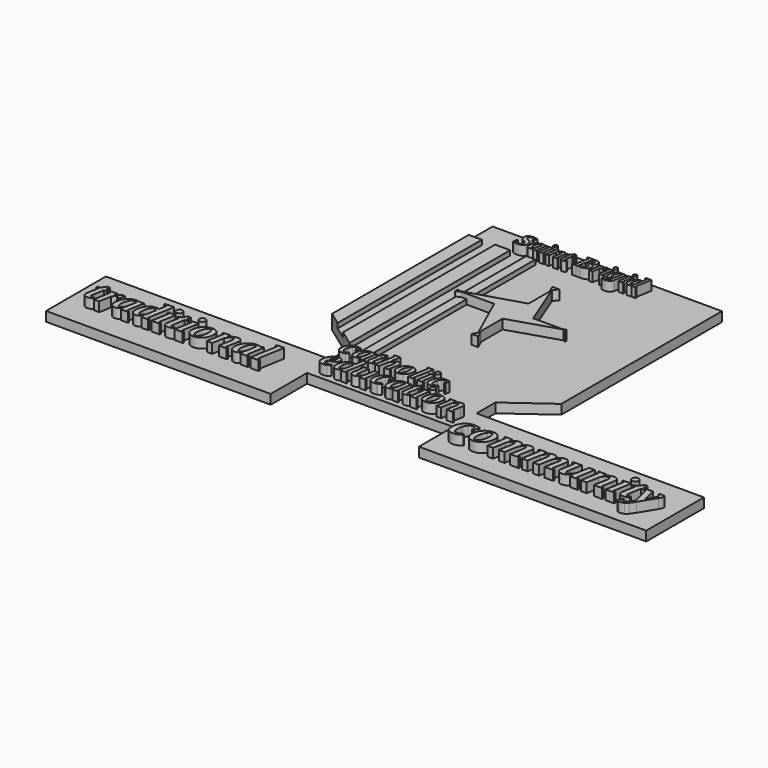
from build123d import *

# Parameters (mm, degrees)
F0_W           = 8.7634572479
F0_H           = 113.4088262916
F0_W_2         = 10.5714052916
F0_H_2         = 19.9463694225
F3_DEPTH       = 6.35
F1_TEXT_SIZE   = 27.5393534038
F1_TEXT_SIZE_2 = 16.523602729
F4_DEPTH       = 12.7
F0_W_3         = 8.7364017963
F0_W_4         = 10.0538036135
F0_W_5         = 6.113210693
F5_DEPTH       = 9.525


# Not quite as in the source:
# - Text() gives the source's letters only with a copy of the font that has no kerning and outlines rounded to 1/6400 em; it was checked with that copy


with BuildPart() as f3:
    # F0 (on Top) → F3 (new body)
    with BuildSketch(Plane.XY):
        Polygon((75.9493485093, 76.8517106771), (-76.2501358986, 76.8517106771), (-76.2501358986, 57.0107996464), (-67.5137341022, 57.0107996464), (-58.7502768544, 57.0107996464), (-48.6964732409, 57.0107996464), (-38.1250679493, 57.0107996464), (-32.0118572563, 57.0107996464), (-25.8986465633, 57.0107996464), (75.9493485093, 57.0107996464), align=None)
        Polygon((75.9493485093, -56.3980266452), (75.9493485093, 57.0107996464), (-25.8986465633, 57.0107996464), (-32.0118572563, 57.0107996464), (-32.0118572563, -56.3980266452), align=None)
        with Locations((-63.1320054783, 0.3063865006)):
            Rectangle(F0_W, F0_H)
        Polygon((48.2921712101, -76.498623082), (75.9493485093, -56.3980266452), (-32.0118572563, -56.3980266452), (-32.0118572563, -76.3443960677), (48.2921712101, -76.3443960677), align=None)
        Polygon((-58.7502768544, -56.3980266452), (-67.5137341022, -56.3980266452), (-67.5137341022, -62.7223944731), (-58.7502768544, -69.0663480104), align=None)
        Polygon((48.2921712101, -92.1651621305), (48.2921712101, -76.498623082), (4.9675871424, -107.9859281933), (48.2921712101, -107.9859281933), align=None)
        Polygon((4.9675871424, -107.9859281933), (48.2921712101, -76.498623082), (48.2921712101, -76.3443960677), (-32.0118572563, -76.3443960677), (-32.0118572563, -88.4225549039), (-4.9872606169, -107.9859281933), align=None)
        with Locations((-43.4107705951, 0.3063865006)):
            Rectangle(F0_W_2, F0_H)
        with Locations((-43.4107705951, -66.3712113564)):
            Rectangle(F0_W_2, F0_H_2)
        Polygon((48.2921712101, -107.9859281933), (4.9675871424, -107.9859281933), (0, -111.5962555718), (48.2921712101, -111.5962555718), align=None)
        Polygon((0, -111.5962555718), (4.9675871424, -107.9859281933), (-4.9872606169, -107.9859281933), align=None)
        Polygon((199.201464653, -92.1651621305), (48.2921712101, -92.1651621305), (48.2921712101, -107.9859281933), (48.2921712101, -111.5962555718), (48.2921712101, -140.0250941515), (199.201464653, -140.0250941515), align=None)
        Polygon((-38.1250679493, -76.3443960677), (-48.6964732409, -76.3443960677), (-38.1250679493, -83.9971411085), align=None)
        Polygon((-38.1250679493, -83.9971411085), (-48.6964732409, -76.3443960677), (-48.6964732409, -92.1651621305), (-48.6964732409, -107.9859281933), (-4.9872606169, -107.9859281933), (-32.0118572563, -88.4225549039), align=None)
        Polygon((-48.6964732409, -111.5962555718), (0, -111.5962555718), (-4.9872606169, -107.9859281933), (-48.6964732409, -107.9859281933), align=None)
        Polygon((-48.6964732409, -107.9859281933), (-48.6964732409, -92.1651621305), (-197.7848261595, -92.1651621305), (-197.7848261595, -141.7777985334), (-48.6964732409, -141.7777985334), (-48.6964732409, -111.5962555718), align=None)
    extrude(amount=F3_DEPTH)

    # F1 (on face) + F2 (on face) → F4 (join)
    with BuildSketch(Plane.XY):
        with BuildLine():
            add(Edge.make_bspline(
                [(-41.3645407825, -91.9325501454), (-43.113672582, -91.9325501454), (-44.0727690147, -90.98645841)],
                knots=[0, 0, 0, 1, 1, 1], degree=2))
            add(Edge.make_bspline(
                [(-39.3683197326, -91.5147742417), (-40.389188478, -91.9325501454), (-41.3645407825, -91.9325501454)],
                knots=[0, 0, 0, 1, 1, 1], degree=2))
            add(Edge.make_bspline(
                [(-37.515150354, -90.3557305865), (-38.3474509872, -91.0969983379), (-39.3683197326, -91.5147742417)],
                knots=[0, 0, 0, 1, 1, 1], degree=2))
            Line((-37.515150354, -90.3557305865), (-37.9605612397, -89.7152492398))
            add(Edge.make_bspline(
                [(-39.1651213358, -90.3963702658), (-38.5392702738, -90.1216460334), (-37.9605612397, -89.7152492398)],
                knots=[0, 0, 0, 1, 1, 1], degree=2))
            add(Edge.make_bspline(
                [(-40.5517471954, -90.6710944982), (-39.7909723979, -90.6710944982), (-39.1651213358, -90.3963702658)],
                knots=[0, 0, 0, 1, 1, 1], degree=2))
            add(Edge.make_bspline(
                [(-41.863596045, -90.0403666747), (-41.4165595721, -90.6710944982), (-40.5517471954, -90.6710944982)],
                knots=[0, 0, 0, 1, 1, 1], degree=2))
            add(Edge.make_bspline(
                [(-42.3106325179, -88.2717278291), (-42.3106325179, -89.4096388511), (-41.863596045, -90.0403666747)],
                knots=[0, 0, 0, 1, 1, 1], degree=2))
            add(Edge.make_bspline(
                [(-41.9042357244, -85.6171439736), (-42.3106325179, -86.8412111158), (-42.3106325179, -88.2717278291)],
                knots=[0, 0, 0, 1, 1, 1], degree=2))
            add(Edge.make_bspline(
                [(-40.780954987, -83.6761928877), (-41.4978389308, -84.3930768315), (-41.9042357244, -85.6171439736)],
                knots=[0, 0, 0, 1, 1, 1], degree=2))
            add(Edge.make_bspline(
                [(-39.2610309791, -82.9593089438), (-40.0640710432, -82.9593089438), (-40.780954987, -83.6761928877)],
                knots=[0, 0, 0, 1, 1, 1], degree=2))
            add(Edge.make_bspline(
                [(-37.7784954762, -83.5705297213), (-38.3279439411, -82.9593089438), (-39.2610309791, -82.9593089438)],
                knots=[0, 0, 0, 1, 1, 1], degree=2))
            Line((-37.7784954762, -83.5705297213), (-37.6354438049, -85.3066568234))
            Line((-37.6354438049, -85.3066568234), (-36.9039295765, -85.3066568234))
            Line((-36.9039295765, -85.3066568234), (-36.4064999012, -82.3805999098))
            add(Edge.make_bspline(
                [(-37.804504871, -82.0603592365), (-36.946194843, -82.1985341463), (-36.4064999012, -82.3805999098)],
                knots=[0, 0, 0, 1, 1, 1], degree=2))
            add(Edge.make_bspline(
                [(-39.3943291274, -81.9221843267), (-38.662814899, -81.9221843267), (-37.804504871, -82.0603592365)],
                knots=[0, 0, 0, 1, 1, 1], degree=2))
            add(Edge.make_bspline(
                [(-42.2293531592, -82.7349779138), (-40.9191298968, -81.9221843267), (-39.3943291274, -81.9221843267)],
                knots=[0, 0, 0, 1, 1, 1], degree=2))
            add(Edge.make_bspline(
                [(-44.2857209346, -85.0221790679), (-43.5395764216, -83.5477715009), (-42.2293531592, -82.7349779138)],
                knots=[0, 0, 0, 1, 1, 1], degree=2))
            add(Edge.make_bspline(
                [(-45.0318654475, -88.3757654083), (-45.0318654475, -86.4965866349), (-44.2857209346, -85.0221790679)],
                knots=[0, 0, 0, 1, 1, 1], degree=2))
            add(Edge.make_bspline(
                [(-44.0727690147, -90.98645841), (-45.0318654475, -90.0403666747), (-45.0318654475, -88.3757654083)],
                knots=[0, 0, 0, 1, 1, 1], degree=2))
        make_face()
        with BuildLine():
            add(Edge.make_bspline(
                [(42.3528729249, -100.0138184269), (42.3528729249, -98.9417919724), (41.3445312103, -98.9417919724)],
                knots=[0, 0, 0, 1, 1, 1], degree=2))
            add(Edge.make_bspline(
                [(42.1087480887, -101.7403824856), (42.3528729249, -100.4560735649), (42.3528729249, -100.0138184269)],
                knots=[0, 0, 0, 1, 1, 1], degree=2))
            Line((42.1087480887, -101.7403824856), (40.9801129766, -108.0310195684))
            Line((40.9801129766, -108.0310195684), (45.2469905479, -108.0310195684))
            Line((45.2469905479, -108.0310195684), (45.3920502332, -107.302183101))
            Line((45.3920502332, -107.302183101), (44.1077413125, -107.0368300182))
            Line((44.1077413125, -107.0368300182), (45.0700884927, -101.616551047))
            add(Edge.make_bspline(
                [(45.3460556989, -99.5963295766), (45.3460556989, -100.1694922355), (45.0700884927, -101.616551047)],
                knots=[0, 0, 0, 1, 1, 1], degree=2))
            add(Edge.make_bspline(
                [(44.705670259, -97.9476024222), (45.3460556989, -98.5349172455), (45.3460556989, -99.5963295766)],
                knots=[0, 0, 0, 1, 1, 1], degree=2))
            add(Edge.make_bspline(
                [(42.9720301181, -97.360287599), (44.0652848192, -97.360287599), (44.705670259, -97.9476024222)],
                knots=[0, 0, 0, 1, 1, 1], degree=2))
            add(Edge.make_bspline(
                [(38.7688372866, -99.5715632889), (40.4812491809, -97.360287599), (42.9720301181, -97.360287599)],
                knots=[0, 0, 0, 1, 1, 1], degree=2))
            Line((38.7688372866, -99.5715632889), (38.8572883142, -97.6362548051))
            Line((38.8572883142, -97.6362548051), (35.1635734017, -97.6362548051))
            Line((35.1635734017, -97.6362548051), (35.0220517576, -98.3686293136))
            Line((35.0220517576, -98.3686293136), (36.0056271844, -98.6445965197))
            Line((36.0056271844, -98.6445965197), (34.3675141533, -108.0310195684))
            Line((34.3675141533, -108.0310195684), (37.3111643518, -108.0310195684))
            Line((37.3111643518, -108.0310195684), (38.4822559572, -101.4644152795))
            add(Edge.make_bspline(
                [(39.7754099807, -99.7166229742), (38.9032828486, -100.4914539759), (38.4822559572, -101.4644152795)],
                knots=[0, 0, 0, 1, 1, 1], degree=2))
            add(Edge.make_bspline(
                [(41.3445312103, -98.9417919724), (40.6475371128, -98.9417919724), (39.7754099807, -99.7166229742)],
                knots=[0, 0, 0, 1, 1, 1], degree=2))
        make_face()
        with BuildLine():
            add(Edge.make_bspline(
                [(60.294291855, -126.8266201223), (57.8249315149, -126.8266201223), (56.4709142281, -125.4909623919)],
                knots=[0, 0, 0, 1, 1, 1], degree=2))
            add(Edge.make_bspline(
                [(63.1124837673, -126.2368193719), (61.6712585874, -126.8266201223), (60.294291855, -126.8266201223)],
                knots=[0, 0, 0, 1, 1, 1], degree=2))
            add(Edge.make_bspline(
                [(65.7287205589, -124.6005239049), (64.5537089472, -125.6470186215), (63.1124837673, -126.2368193719)],
                knots=[0, 0, 0, 1, 1, 1], degree=2))
            Line((65.7287205589, -124.6005239049), (65.0999057511, -123.6963157506))
            add(Edge.make_bspline(
                [(63.3993518366, -124.6578975188), (64.2829054899, -124.2700518891), (65.0999057511, -123.6963157506)],
                knots=[0, 0, 0, 1, 1, 1], degree=2))
            add(Edge.make_bspline(
                [(61.441764132, -125.0457431484), (62.5157981833, -125.0457431484), (63.3993518366, -124.6578975188)],
                knots=[0, 0, 0, 1, 1, 1], degree=2))
            add(Edge.make_bspline(
                [(59.5897438769, -124.1553046614), (60.2208536293, -125.0457431484), (61.441764132, -125.0457431484)],
                knots=[0, 0, 0, 1, 1, 1], degree=2))
            add(Edge.make_bspline(
                [(58.9586341246, -121.6584049867), (58.9586341246, -123.2648661745), (59.5897438769, -124.1553046614)],
                knots=[0, 0, 0, 1, 1, 1], degree=2))
            add(Edge.make_bspline(
                [(59.5323702631, -117.91076053), (58.9586341246, -119.6388537792), (58.9586341246, -121.6584049867)],
                knots=[0, 0, 0, 1, 1, 1], degree=2))
            add(Edge.make_bspline(
                [(61.1181769499, -115.1705967325), (60.1061064016, -116.1826672809), (59.5323702631, -117.91076053)],
                knots=[0, 0, 0, 1, 1, 1], degree=2))
            add(Edge.make_bspline(
                [(63.2639501079, -114.1585261842), (62.1302474982, -114.1585261842), (61.1181769499, -115.1705967325)],
                knots=[0, 0, 0, 1, 1, 1], degree=2))
            add(Edge.make_bspline(
                [(65.3569395411, -115.0214253365), (64.5812482819, -114.1585261842), (63.2639501079, -114.1585261842)],
                knots=[0, 0, 0, 1, 1, 1], degree=2))
            Line((65.3569395411, -115.0214253365), (65.5588946619, -117.4724261202))
            Line((65.5588946619, -117.4724261202), (66.5916197112, -117.4724261202))
            Line((66.5916197112, -117.4724261202), (67.2938727447, -113.341525923))
            add(Edge.make_bspline(
                [(65.3202204283, -112.8894218459), (66.5319511528, -113.084492133), (67.2938727447, -113.341525923)],
                knots=[0, 0, 0, 1, 1, 1], degree=2))
            add(Edge.make_bspline(
                [(63.0757646545, -112.6943515588), (64.1084897038, -112.6943515588), (65.3202204283, -112.8894218459)],
                knots=[0, 0, 0, 1, 1, 1], degree=2))
            add(Edge.make_bspline(
                [(59.0733813523, -113.8418238358), (60.9231066628, -112.6943515588), (63.0757646545, -112.6943515588)],
                knots=[0, 0, 0, 1, 1, 1], degree=2))
            add(Edge.make_bspline(
                [(56.1702764915, -117.0708108233), (57.2236560418, -114.9892961128), (59.0733813523, -113.8418238358)],
                knots=[0, 0, 0, 1, 1, 1], degree=2))
            add(Edge.make_bspline(
                [(55.1168969412, -121.8052814382), (55.1168969412, -119.1523255337), (56.1702764915, -117.0708108233)],
                knots=[0, 0, 0, 1, 1, 1], degree=2))
            add(Edge.make_bspline(
                [(56.4709142281, -125.4909623919), (55.1168969412, -124.1553046614), (55.1168969412, -121.8052814382)],
                knots=[0, 0, 0, 1, 1, 1], degree=2))
        make_face()
        with BuildLine():
            add(Edge.make_bspline(
                [(99.9142146352, -116.1367683898), (99.9142146352, -114.7460319901), (98.8814895859, -114.7460319901)],
                knots=[0, 0, 0, 1, 1, 1], degree=2))
            add(Edge.make_bspline(
                [(99.5975122868, -118.3766342745), (99.9142146352, -116.7105045283), (99.9142146352, -116.1367683898)],
                knots=[0, 0, 0, 1, 1, 1], degree=2))
            Line((99.5975122868, -118.3766342745), (98.1333376613, -126.5374571085))
            Line((98.1333376613, -126.5374571085), (103.6687439256, -126.5374571085))
            Line((103.6687439256, -126.5374571085), (103.856929379, -125.5919399523))
            Line((103.856929379, -125.5919399523), (102.1907996328, -125.2476982692))
            Line((102.1907996328, -125.2476982692), (103.5539966979, -117.6147126826))
            add(Edge.make_bspline(
                [(103.7972608206, -115.7236783701), (103.7972608206, -116.2515156175), (103.5539966979, -117.6147126826)],
                knots=[0, 0, 0, 1, 1, 1], degree=2))
            add(Edge.make_bspline(
                [(103.0514038406, -113.490697319), (103.7972608206, -114.2870430793), (103.7972608206, -115.7236783701)],
                knots=[0, 0, 0, 1, 1, 1], degree=2))
            add(Edge.make_bspline(
                [(101.0433273558, -112.6943515588), (102.3055468605, -112.6943515588), (103.0514038406, -113.490697319)],
                knots=[0, 0, 0, 1, 1, 1], degree=2))
            add(Edge.make_bspline(
                [(96.1964044578, -115.5354929166), (98.2205455544, -112.6943515588), (101.0433273558, -112.6943515588)],
                knots=[0, 0, 0, 1, 1, 1], degree=2))
            add(Edge.make_bspline(
                [(95.4574323114, -113.4470933725), (96.1826347904, -114.1998351862), (96.1964044578, -115.5354929166)],
                knots=[0, 0, 0, 1, 1, 1], degree=2))
            add(Edge.make_bspline(
                [(93.4562406603, -112.6943515588), (94.7322298323, -112.6943515588), (95.4574323114, -113.4470933725)],
                knots=[0, 0, 0, 1, 1, 1], degree=2))
            add(Edge.make_bspline(
                [(90.8629533143, -113.3759500913), (92.0241952586, -112.6943515588), (93.4562406603, -112.6943515588)],
                knots=[0, 0, 0, 1, 1, 1], degree=2))
            add(Edge.make_bspline(
                [(88.6689863207, -115.4620546909), (89.70171137, -114.0575486239), (90.8629533143, -113.3759500913)],
                knots=[0, 0, 0, 1, 1, 1], degree=2))
            Line((88.6689863207, -115.4620546909), (88.7102953226, -113.0523629092))
            Line((88.7102953226, -113.0523629092), (84.0056589869, -113.0523629092))
            Line((84.0056589869, -113.0523629092), (83.8174735335, -114.0024699546))
            Line((83.8174735335, -114.0024699546), (85.0934627055, -114.360481305))
            Line((85.0934627055, -114.360481305), (82.9729339376, -126.5374571085))
            Line((82.9729339376, -126.5374571085), (86.7871317864, -126.5374571085))
            Line((86.7871317864, -126.5374571085), (88.3063850811, -118.0186229241))
            add(Edge.make_bspline(
                [(89.6994164254, -115.7007289245), (88.8250425503, -116.655425859), (88.3063850811, -118.0186229241)],
                knots=[0, 0, 0, 1, 1, 1], degree=2))
            add(Edge.make_bspline(
                [(91.2622736667, -114.7460319901), (90.5737903005, -114.7460319901), (89.6994164254, -115.7007289245)],
                knots=[0, 0, 0, 1, 1, 1], degree=2))
            add(Edge.make_bspline(
                [(92.3225380506, -116.1367683898), (92.3225380506, -114.7460319901), (91.2622736667, -114.7460319901)],
                knots=[0, 0, 0, 1, 1, 1], degree=2))
            add(Edge.make_bspline(
                [(92.0104255913, -118.3766342745), (92.3225380506, -116.7105045283), (92.3225380506, -116.1367683898)],
                knots=[0, 0, 0, 1, 1, 1], degree=2))
            Line((92.0104255913, -118.3766342745), (90.5462509658, -126.5374571085))
            Line((90.5462509658, -126.5374571085), (94.3742184819, -126.5374571085))
            Line((94.3742184819, -126.5374571085), (95.7970841054, -118.4638421675))
            add(Edge.make_bspline(
                [(96.4763876934, -116.783942754), (95.9393706677, -117.674381241), (95.7970841054, -118.4638421675)],
                knots=[0, 0, 0, 1, 1, 1], degree=2))
            add(Edge.make_bspline(
                [(97.6950032515, -115.3197681286), (97.013404719, -115.8935042671), (96.4763876934, -116.783942754)],
                knots=[0, 0, 0, 1, 1, 1], degree=2))
            add(Edge.make_bspline(
                [(98.8814895859, -114.7460319901), (98.3766017841, -114.7460319901), (97.6950032515, -115.3197681286)],
                knots=[0, 0, 0, 1, 1, 1], degree=2))
        make_face()
        with BuildLine():
            add(Edge.make_bspline(
                [(122.7626826148, -116.1367683898), (122.7626826148, -114.7460319901), (121.7299575655, -114.7460319901)],
                knots=[0, 0, 0, 1, 1, 1], degree=2))
            add(Edge.make_bspline(
                [(122.4459802664, -118.3766342745), (122.7626826148, -116.7105045283), (122.7626826148, -116.1367683898)],
                knots=[0, 0, 0, 1, 1, 1], degree=2))
            Line((122.4459802664, -118.3766342745), (120.9818056409, -126.5374571085))
            Line((120.9818056409, -126.5374571085), (126.5172119052, -126.5374571085))
            Line((126.5172119052, -126.5374571085), (126.7053973586, -125.5919399523))
            Line((126.7053973586, -125.5919399523), (125.0392676124, -125.2476982692))
            Line((125.0392676124, -125.2476982692), (126.4024646775, -117.6147126826))
            add(Edge.make_bspline(
                [(126.6457288002, -115.7236783701), (126.6457288002, -116.2515156175), (126.4024646775, -117.6147126826)],
                knots=[0, 0, 0, 1, 1, 1], degree=2))
            add(Edge.make_bspline(
                [(125.8998718202, -113.490697319), (126.6457288002, -114.2870430793), (126.6457288002, -115.7236783701)],
                knots=[0, 0, 0, 1, 1, 1], degree=2))
            add(Edge.make_bspline(
                [(123.8917953354, -112.6943515588), (125.1540148401, -112.6943515588), (125.8998718202, -113.490697319)],
                knots=[0, 0, 0, 1, 1, 1], degree=2))
            add(Edge.make_bspline(
                [(119.0448724374, -115.5354929166), (121.069013534, -112.6943515588), (123.8917953354, -112.6943515588)],
                knots=[0, 0, 0, 1, 1, 1], degree=2))
            add(Edge.make_bspline(
                [(118.305900291, -113.4470933725), (119.03110277, -114.1998351862), (119.0448724374, -115.5354929166)],
                knots=[0, 0, 0, 1, 1, 1], degree=2))
            add(Edge.make_bspline(
                [(116.3047086399, -112.6943515588), (117.5806978119, -112.6943515588), (118.305900291, -113.4470933725)],
                knots=[0, 0, 0, 1, 1, 1], degree=2))
            add(Edge.make_bspline(
                [(113.7114212939, -113.3759500913), (114.8726632382, -112.6943515588), (116.3047086399, -112.6943515588)],
                knots=[0, 0, 0, 1, 1, 1], degree=2))
            add(Edge.make_bspline(
                [(111.5174543003, -115.4620546909), (112.5501793496, -114.0575486239), (113.7114212939, -113.3759500913)],
                knots=[0, 0, 0, 1, 1, 1], degree=2))
            Line((111.5174543003, -115.4620546909), (111.5587633022, -113.0523629092))
            Line((111.5587633022, -113.0523629092), (106.8541269665, -113.0523629092))
            Line((106.8541269665, -113.0523629092), (106.6659415131, -114.0024699546))
            Line((106.6659415131, -114.0024699546), (107.9419306851, -114.360481305))
            Line((107.9419306851, -114.360481305), (105.8214019172, -126.5374571085))
            Line((105.8214019172, -126.5374571085), (109.635599766, -126.5374571085))
            Line((109.635599766, -126.5374571085), (111.1548530607, -118.0186229241))
            add(Edge.make_bspline(
                [(112.547884405, -115.7007289245), (111.6735105299, -116.655425859), (111.1548530607, -118.0186229241)],
                knots=[0, 0, 0, 1, 1, 1], degree=2))
            add(Edge.make_bspline(
                [(114.1107416463, -114.7460319901), (113.4222582801, -114.7460319901), (112.547884405, -115.7007289245)],
                knots=[0, 0, 0, 1, 1, 1], degree=2))
            add(Edge.make_bspline(
                [(115.1710060302, -116.1367683898), (115.1710060302, -114.7460319901), (114.1107416463, -114.7460319901)],
                knots=[0, 0, 0, 1, 1, 1], degree=2))
            add(Edge.make_bspline(
                [(114.8588935709, -118.3766342745), (115.1710060302, -116.7105045283), (115.1710060302, -116.1367683898)],
                knots=[0, 0, 0, 1, 1, 1], degree=2))
            Line((114.8588935709, -118.3766342745), (113.3947189454, -126.5374571085))
            Line((113.3947189454, -126.5374571085), (117.2226864615, -126.5374571085))
            Line((117.2226864615, -126.5374571085), (118.645552085, -118.4638421675))
            add(Edge.make_bspline(
                [(119.324855673, -116.783942754), (118.7878386473, -117.674381241), (118.645552085, -118.4638421675)],
                knots=[0, 0, 0, 1, 1, 1], degree=2))
            add(Edge.make_bspline(
                [(120.5434712311, -115.3197681286), (119.8618726986, -115.8935042671), (119.324855673, -116.783942754)],
                knots=[0, 0, 0, 1, 1, 1], degree=2))
            add(Edge.make_bspline(
                [(121.7299575655, -114.7460319901), (121.2250697637, -114.7460319901), (120.5434712311, -115.3197681286)],
                knots=[0, 0, 0, 1, 1, 1], degree=2))
        make_face()
        with BuildLine():
            add(Edge.make_bspline(
                [(133.1312421098, -123.4392819606), (133.1312421098, -124.8300183603), (134.4347706165, -124.8300183603)],
                knots=[0, 0, 0, 1, 1, 1], degree=2))
            add(Edge.make_bspline(
                [(133.4479444583, -121.1994160759), (133.1312421098, -122.8517761548), (133.1312421098, -123.4392819606)],
                knots=[0, 0, 0, 1, 1, 1], degree=2))
            Line((133.4479444583, -121.1994160759), (134.9075291946, -113.0523629092))
            Line((134.9075291946, -113.0523629092), (129.3721229304, -113.0523629092))
            Line((129.3721229304, -113.0523629092), (129.1839374769, -114.0024699546))
            Line((129.1839374769, -114.0024699546), (130.8500672231, -114.3467116377))
            add(Edge.make_bspline(
                [(129.3376987621, -122.922919436), (129.4317914888, -122.264270349), (130.8500672231, -114.3467116377)],
                knots=[0, 0, 0, 1, 1, 1], degree=2))
            add(Edge.make_bspline(
                [(129.2436060353, -123.8569618694), (129.2436060353, -123.5815685229), (129.3376987621, -122.922919436)],
                knots=[0, 0, 0, 1, 1, 1], degree=2))
            add(Edge.make_bspline(
                [(130.0606062966, -126.0991226987), (129.2436060353, -125.3165466058), (129.2436060353, -123.8569618694)],
                knots=[0, 0, 0, 1, 1, 1], degree=2))
            add(Edge.make_bspline(
                [(132.3280115159, -126.8816987916), (130.8776065578, -126.8816987916), (130.0606062966, -126.0991226987)],
                knots=[0, 0, 0, 1, 1, 1], degree=2))
            add(Edge.make_bspline(
                [(137.7762098871, -124.0130180991), (135.5547035588, -126.8816987916), (132.3280115159, -126.8816987916)],
                knots=[0, 0, 0, 1, 1, 1], degree=2))
            Line((137.7762098871, -124.0130180991), (137.6614626594, -126.5374571085))
            Line((137.6614626594, -126.5374571085), (142.742469902, -126.5374571085))
            Line((142.742469902, -126.5374571085), (142.9260654663, -125.5919399523))
            Line((142.9260654663, -125.5919399523), (141.3655031696, -125.2339286018))
            Line((141.3655031696, -125.2339286018), (143.4860319375, -113.0523629092))
            Line((143.4860319375, -113.0523629092), (139.6718340887, -113.0523629092))
            Line((139.6718340887, -113.0523629092), (138.152580794, -121.5620173154))
            add(Edge.make_bspline(
                [(136.5002207151, -123.8041781447), (137.6476929921, -122.778337929), (138.152580794, -121.5620173154)],
                knots=[0, 0, 0, 1, 1, 1], degree=2))
            add(Edge.make_bspline(
                [(134.4347706165, -124.8300183603), (135.3527484381, -124.8300183603), (136.5002207151, -123.8041781447)],
                knots=[0, 0, 0, 1, 1, 1], degree=2))
        make_face()
        with BuildLine():
            add(Edge.make_bspline(
                [(155.4059739509, -116.1367683898), (155.4059739509, -114.7460319901), (154.0978555551, -114.7460319901)],
                knots=[0, 0, 0, 1, 1, 1], degree=2))
            add(Edge.make_bspline(
                [(155.0892716025, -118.3766342745), (155.4059739509, -116.7105045283), (155.4059739509, -116.1367683898)],
                knots=[0, 0, 0, 1, 1, 1], degree=2))
            Line((155.0892716025, -118.3766342745), (153.625096977, -126.5374571085))
            Line((153.625096977, -126.5374571085), (159.1605032413, -126.5374571085))
            Line((159.1605032413, -126.5374571085), (159.3486886947, -125.5919399523))
            Line((159.3486886947, -125.5919399523), (157.6825589485, -125.2476982692))
            Line((157.6825589485, -125.2476982692), (158.9310087859, -118.2159881557))
            add(Edge.make_bspline(
                [(159.2890201363, -115.595161475), (159.2890201363, -116.3387235105), (158.9310087859, -118.2159881557)],
                knots=[0, 0, 0, 1, 1, 1], degree=2))
            add(Edge.make_bspline(
                [(158.4582502077, -113.4562731507), (159.2890201363, -114.2181947426), (159.2890201363, -115.595161475)],
                knots=[0, 0, 0, 1, 1, 1], degree=2))
            add(Edge.make_bspline(
                [(156.2092045448, -112.6943515588), (157.6274802792, -112.6943515588), (158.4582502077, -113.4562731507)],
                knots=[0, 0, 0, 1, 1, 1], degree=2))
            add(Edge.make_bspline(
                [(150.7564162845, -115.5630322513), (152.9779226128, -112.6943515588), (156.2092045448, -112.6943515588)],
                knots=[0, 0, 0, 1, 1, 1], degree=2))
            Line((150.7564162845, -115.5630322513), (150.8711635122, -113.0523629092))
            Line((150.8711635122, -113.0523629092), (146.0793192835, -113.0523629092))
            Line((146.0793192835, -113.0523629092), (145.8957237191, -114.0024699546))
            Line((145.8957237191, -114.0024699546), (147.1717128912, -114.360481305))
            Line((147.1717128912, -114.360481305), (145.0465942342, -126.5374571085))
            Line((145.0465942342, -126.5374571085), (148.865381972, -126.5374571085))
            Line((148.865381972, -126.5374571085), (150.3846352668, -118.0186229241))
            add(Edge.make_bspline(
                [(152.0622397357, -115.7512177047), (150.9308320706, -116.7564034194), (150.3846352668, -118.0186229241)],
                knots=[0, 0, 0, 1, 1, 1], degree=2))
            add(Edge.make_bspline(
                [(154.0978555551, -114.7460319901), (153.1936474009, -114.7460319901), (152.0622397357, -115.7512177047)],
                knots=[0, 0, 0, 1, 1, 1], degree=2))
        make_face()
        Polygon((167.3213260753, -125.5919399523), (165.6138873271, -125.2476982692), (167.7665453188, -113.0523629092), (162.5294818465, -113.0523629092), (162.3734256169, -114.0024699546), (163.6769541235, -114.3467116377), (161.528886021, -126.5374571085), (167.1652698456, -126.5374571085), align=None)
        with BuildLine():
            add(Edge.make_bspline(
                [(164.4113363808, -108.3477265735), (164.4113363808, -107.4159790846), (165.0631006341, -106.7848693322)],
                knots=[0, 0, 0, 1, 1, 1], degree=2))
            add(Edge.make_bspline(
                [(165.0562158005, -109.9220585376), (164.4113363808, -109.2840639515), (164.4113363808, -108.3477265735)],
                knots=[0, 0, 0, 1, 1, 1], degree=2))
            add(Edge.make_bspline(
                [(166.6190730418, -110.5600531236), (165.7010952202, -110.5600531236), (165.0562158005, -109.9220585376)],
                knots=[0, 0, 0, 1, 1, 1], degree=2))
            add(Edge.make_bspline(
                [(168.181930283, -109.9059939257), (167.5508205307, -110.5600531236), (166.6190730418, -110.5600531236)],
                knots=[0, 0, 0, 1, 1, 1], degree=2))
            add(Edge.make_bspline(
                [(168.8130400354, -108.3477265735), (168.8130400354, -109.2519347278), (168.181930283, -109.9059939257)],
                knots=[0, 0, 0, 1, 1, 1], degree=2))
            add(Edge.make_bspline(
                [(168.1750454494, -106.7917541659), (168.8130400354, -107.4297487519), (168.8130400354, -108.3477265735)],
                knots=[0, 0, 0, 1, 1, 1], degree=2))
            add(Edge.make_bspline(
                [(166.6190730418, -106.1537595799), (167.5370508634, -106.1537595799), (168.1750454494, -106.7917541659)],
                knots=[0, 0, 0, 1, 1, 1], degree=2))
            add(Edge.make_bspline(
                [(165.0631006341, -106.7848693322), (165.7148648875, -106.1537595799), (166.6190730418, -106.1537595799)],
                knots=[0, 0, 0, 1, 1, 1], degree=2))
        make_face()
        with BuildLine():
            add(Edge.make_bspline(
                [(-21.3470603194, -90.6515874522), (-21.0024358385, -90.6515874522), (-20.2319075179, -90.3849911556)],
                knots=[0, 0, 0, 1, 1, 1], degree=2))
            add(Edge.make_bspline(
                [(-22.0037975378, -90.407749376), (-21.7339500668, -90.6515874522), (-21.3470603194, -90.6515874522)],
                knots=[0, 0, 0, 1, 1, 1], degree=2))
            add(Edge.make_bspline(
                [(-22.2736450087, -89.6242163581), (-22.2736450087, -90.1639112999), (-22.0037975378, -90.407749376)],
                knots=[0, 0, 0, 1, 1, 1], degree=2))
            add(Edge.make_bspline(
                [(-22.1110862913, -88.4050259774), (-22.2736450087, -89.2373266106), (-22.2736450087, -89.6242163581)],
                knots=[0, 0, 0, 1, 1, 1], degree=2))
            Line((-22.1110862913, -88.4050259774), (-21.184501602, -83.2324075891))
            Line((-21.184501602, -83.2324075891), (-19.5816726482, -83.2324075891))
            Line((-19.5816726482, -83.2324075891), (-19.3963557103, -82.1757759259))
            Line((-19.3963557103, -82.1757759259), (-21.0024358385, -82.1757759259))
            Line((-21.0024358385, -82.1757759259), (-20.615546091, -80.0137449842))
            Line((-20.615546091, -80.0137449842), (-22.1013327682, -80.0137449842))
            Line((-22.1013327682, -80.0137449842), (-23.5123424354, -82.1757759259))
            Line((-23.5123424354, -82.1757759259), (-24.9558638461, -82.5724191964))
            Line((-24.9558638461, -82.5724191964), (-25.066403774, -83.2324075891))
            Line((-25.066403774, -83.2324075891), (-23.8992321829, -83.2324075891))
            Line((-23.8992321829, -83.2324075891), (-24.8323192209, -88.3855189313))
            add(Edge.make_bspline(
                [(-25.0176361587, -89.8485473881), (-25.0176361587, -89.3803782819), (-24.8323192209, -88.3855189313)],
                knots=[0, 0, 0, 1, 1, 1], degree=2))
            add(Edge.make_bspline(
                [(-24.4129177299, -91.3977319651), (-25.0176361587, -90.8629137848), (-25.0176361587, -89.8485473881)],
                knots=[0, 0, 0, 1, 1, 1], degree=2))
            add(Edge.make_bspline(
                [(-22.6897953253, -91.9325501454), (-23.8081993011, -91.9325501454), (-24.4129177299, -91.3977319651)],
                knots=[0, 0, 0, 1, 1, 1], degree=2))
            add(Edge.make_bspline(
                [(-21.23164363, -91.6935888308), (-21.9972951891, -91.9325501454), (-22.6897953253, -91.9325501454)],
                knots=[0, 0, 0, 1, 1, 1], degree=2))
            add(Edge.make_bspline(
                [(-19.9653112213, -91.0969983379), (-20.465992071, -91.4546275162), (-21.23164363, -91.6935888308)],
                knots=[0, 0, 0, 1, 1, 1], degree=2))
            Line((-19.9653112213, -91.0969983379), (-20.2319075179, -90.3849911556))
        make_face()
        with BuildLine():
            add(Edge.make_bspline(
                [(-15.4851929692, -83.9151542023), (-13.9213781076, -81.9221843267), (-11.6065419716, -81.9221843267)],
                knots=[0, 0, 0, 1, 1, 1], degree=2))
            Line((-15.4851929692, -83.9151542023), (-15.4169183079, -83.6192973366))
            Line((-15.4169183079, -83.6192973366), (-15.0918008731, -81.9937101624))
            Line((-15.0918008731, -81.9937101624), (-14.2367420194, -77.2892608802))
            Line((-14.2367420194, -77.2892608802), (-17.946331951, -77.2892608802))
            Line((-17.946331951, -77.2892608802), (-18.0568718788, -77.9622539703))
            Line((-18.0568718788, -77.9622539703), (-17.1335383639, -78.2060920465))
            Line((-17.1335383639, -78.2060920465), (-19.5101468125, -91.7277261615))
            Line((-19.5101468125, -91.7277261615), (-16.808420929, -91.7277261615))
            Line((-16.808420929, -91.7277261615), (-15.7290310453, -85.6935465708))
            add(Edge.make_bspline(
                [(-14.5423524082, -84.0874664427), (-15.3453924722, -84.799473625), (-15.7290310453, -85.6935465708)],
                knots=[0, 0, 0, 1, 1, 1], degree=2))
            add(Edge.make_bspline(
                [(-13.0988309975, -83.3754592604), (-13.7393123441, -83.3754592604), (-14.5423524082, -84.0874664427)],
                knots=[0, 0, 0, 1, 1, 1], degree=2))
            add(Edge.make_bspline(
                [(-12.1754974825, -84.360565088), (-12.1754974825, -83.3754592604), (-13.0988309975, -83.3754592604)],
                knots=[0, 0, 0, 1, 1, 1], degree=2))
            add(Edge.make_bspline(
                [(-12.3965773382, -85.94713817), (-12.1754974825, -84.7669618815), (-12.1754974825, -84.360565088)],
                knots=[0, 0, 0, 1, 1, 1], degree=2))
            Line((-12.3965773382, -85.94713817), (-13.4337019554, -91.7277261615))
            Line((-13.4337019554, -91.7277261615), (-9.5127856912, -91.7277261615))
            Line((-9.5127856912, -91.7277261615), (-9.3794875429, -91.0579842457))
            Line((-9.3794875429, -91.0579842457), (-10.5596638314, -90.8141461696))
            Line((-10.5596638314, -90.8141461696), (-9.5940650499, -85.4171967512))
            add(Edge.make_bspline(
                [(-9.4217528094, -83.9444147714), (-9.4217528094, -84.4743561902), (-9.5940650499, -85.4171967512)],
                knots=[0, 0, 0, 1, 1, 1], degree=2))
            add(Edge.make_bspline(
                [(-10.0215944767, -82.46675603), (-9.4217528094, -83.0113277334), (-9.4217528094, -83.9444147714)],
                knots=[0, 0, 0, 1, 1, 1], degree=2))
            add(Edge.make_bspline(
                [(-11.6065419716, -81.9221843267), (-10.621436144, -81.9221843267), (-10.0215944767, -82.46675603)],
                knots=[0, 0, 0, 1, 1, 1], degree=2))
        make_face()
        Polygon((6.6195414256, -91.0579842457), (5.410104568, -90.8141461696), (7.8094712371, -77.2892608802), (4.0998813056, -77.2892608802), (3.9893413777, -77.9622539703), (4.9126748927, -78.2060920465), (2.5165593979, -91.7277261615), (6.5090014978, -91.7277261615), align=None)
        Polygon((12.4716552527, -91.0579842457), (11.2622183951, -90.8141461696), (12.7870191645, -82.1757759259), (9.077429233, -82.1757759259), (8.9668893052, -82.848769016), (9.8902228201, -83.0926070921), (8.368673225, -91.7277261615), (12.3611153249, -91.7277261615), align=None)
        with BuildLine():
            add(Edge.make_bspline(
                [(10.4104107158, -78.8433222187), (10.4104107158, -78.183333826), (10.8720774733, -77.7362973531)],
                knots=[0, 0, 0, 1, 1, 1], degree=2))
            add(Edge.make_bspline(
                [(10.8672007118, -79.9584750202), (10.4104107158, -79.5065617858), (10.4104107158, -78.8433222187)],
                knots=[0, 0, 0, 1, 1, 1], degree=2))
            add(Edge.make_bspline(
                [(11.9742255774, -80.4103882547), (11.3239907078, -80.4103882547), (10.8672007118, -79.9584750202)],
                knots=[0, 0, 0, 1, 1, 1], degree=2))
            add(Edge.make_bspline(
                [(13.0812504431, -79.94709591), (12.6342139702, -80.4103882547), (11.9742255774, -80.4103882547)],
                knots=[0, 0, 0, 1, 1, 1], degree=2))
            add(Edge.make_bspline(
                [(13.528286916, -78.8433222187), (13.528286916, -79.4838035654), (13.0812504431, -79.94709591)],
                knots=[0, 0, 0, 1, 1, 1], degree=2))
            add(Edge.make_bspline(
                [(13.0763736815, -77.7411741146), (13.528286916, -78.1930873491), (13.528286916, -78.8433222187)],
                knots=[0, 0, 0, 1, 1, 1], degree=2))
            add(Edge.make_bspline(
                [(11.9742255774, -77.2892608802), (12.6244604471, -77.2892608802), (13.0763736815, -77.7411741146)],
                knots=[0, 0, 0, 1, 1, 1], degree=2))
            add(Edge.make_bspline(
                [(10.8720774733, -77.7362973531), (11.3337442308, -77.2892608802), (11.9742255774, -77.2892608802)],
                knots=[0, 0, 0, 1, 1, 1], degree=2))
        make_face()
        with BuildLine():
            add(Edge.make_bspline(
                [(17.5922548515, -91.9325501454), (15.843123052, -91.9325501454), (14.8840266193, -90.98645841)],
                knots=[0, 0, 0, 1, 1, 1], degree=2))
            add(Edge.make_bspline(
                [(19.5884759014, -91.5147742417), (18.567607156, -91.9325501454), (17.5922548515, -91.9325501454)],
                knots=[0, 0, 0, 1, 1, 1], degree=2))
            add(Edge.make_bspline(
                [(21.44164528, -90.3557305865), (20.6093446468, -91.0969983379), (19.5884759014, -91.5147742417)],
                knots=[0, 0, 0, 1, 1, 1], degree=2))
            Line((21.44164528, -90.3557305865), (20.9962343943, -89.7152492398))
            add(Edge.make_bspline(
                [(19.7916742982, -90.3963702658), (20.4175253602, -90.1216460334), (20.9962343943, -89.7152492398)],
                knots=[0, 0, 0, 1, 1, 1], degree=2))
            add(Edge.make_bspline(
                [(18.4050484386, -90.6710944982), (19.1658232361, -90.6710944982), (19.7916742982, -90.3963702658)],
                knots=[0, 0, 0, 1, 1, 1], degree=2))
            add(Edge.make_bspline(
                [(17.093199589, -90.0403666747), (17.5402360619, -90.6710944982), (18.4050484386, -90.6710944982)],
                knots=[0, 0, 0, 1, 1, 1], degree=2))
            add(Edge.make_bspline(
                [(16.6461631161, -88.2717278291), (16.6461631161, -89.4096388511), (17.093199589, -90.0403666747)],
                knots=[0, 0, 0, 1, 1, 1], degree=2))
            add(Edge.make_bspline(
                [(17.0525599096, -85.6171439736), (16.6461631161, -86.8412111158), (16.6461631161, -88.2717278291)],
                knots=[0, 0, 0, 1, 1, 1], degree=2))
            add(Edge.make_bspline(
                [(18.175840647, -83.6761928877), (17.4589567032, -84.3930768315), (17.0525599096, -85.6171439736)],
                knots=[0, 0, 0, 1, 1, 1], degree=2))
            add(Edge.make_bspline(
                [(19.6957646549, -82.9593089438), (18.8927245908, -82.9593089438), (18.175840647, -83.6761928877)],
                knots=[0, 0, 0, 1, 1, 1], degree=2))
            add(Edge.make_bspline(
                [(21.1783001578, -83.5705297213), (20.6288516929, -82.9593089438), (19.6957646549, -82.9593089438)],
                knots=[0, 0, 0, 1, 1, 1], degree=2))
            Line((21.1783001578, -83.5705297213), (21.3213518291, -85.3066568234))
            Line((21.3213518291, -85.3066568234), (22.0528660575, -85.3066568234))
            Line((22.0528660575, -85.3066568234), (22.5502957328, -82.3805999098))
            add(Edge.make_bspline(
                [(21.152290763, -82.0603592365), (22.010600791, -82.1985341463), (22.5502957328, -82.3805999098)],
                knots=[0, 0, 0, 1, 1, 1], degree=2))
            add(Edge.make_bspline(
                [(19.5624665066, -81.9221843267), (20.293980735, -81.9221843267), (21.152290763, -82.0603592365)],
                knots=[0, 0, 0, 1, 1, 1], degree=2))
            add(Edge.make_bspline(
                [(16.7274424748, -82.7349779138), (18.0376657372, -81.9221843267), (19.5624665066, -81.9221843267)],
                knots=[0, 0, 0, 1, 1, 1], degree=2))
            add(Edge.make_bspline(
                [(14.6710746994, -85.0221790679), (15.4172192124, -83.5477715009), (16.7274424748, -82.7349779138)],
                knots=[0, 0, 0, 1, 1, 1], degree=2))
            add(Edge.make_bspline(
                [(13.9249301865, -88.3757654083), (13.9249301865, -86.4965866349), (14.6710746994, -85.0221790679)],
                knots=[0, 0, 0, 1, 1, 1], degree=2))
            add(Edge.make_bspline(
                [(14.8840266193, -90.98645841), (13.9249301865, -90.0403666747), (13.9249301865, -88.3757654083)],
                knots=[0, 0, 0, 1, 1, 1], degree=2))
        make_face()
        with BuildLine():
            add(Edge.make_bspline(
                [(-35.7847648556, -99.6281719466), (-35.7847648556, -100.6223614968), (-36.513601323, -101.462646259)],
                knots=[0, 0, 0, 1, 1, 1], degree=2))
            add(Edge.make_bspline(
                [(-36.6851963166, -97.9741377305), (-35.7847648556, -98.587987862), (-35.7847648556, -99.6281719466)],
                knots=[0, 0, 0, 1, 1, 1], degree=2))
            add(Edge.make_bspline(
                [(-39.1140615344, -97.360287599), (-37.5856277775, -97.360287599), (-36.6851963166, -97.9741377305)],
                knots=[0, 0, 0, 1, 1, 1], degree=2))
            add(Edge.make_bspline(
                [(-41.8666575133, -98.2943304504), (-40.5398920993, -97.360287599), (-39.1140615344, -97.360287599)],
                knots=[0, 0, 0, 1, 1, 1], degree=2))
            add(Edge.make_bspline(
                [(-44.000096299, -100.8541031891), (-43.1934229273, -99.2283733018), (-41.8666575133, -98.2943304504)],
                knots=[0, 0, 0, 1, 1, 1], degree=2))
            add(Edge.make_bspline(
                [(-44.8067696707, -104.3815301697), (-44.8067696707, -102.4798330764), (-44.000096299, -100.8541031891)],
                knots=[0, 0, 0, 1, 1, 1], degree=2))
            add(Edge.make_bspline(
                [(-43.77896873, -107.2685717105), (-44.8067696707, -106.2832272631), (-44.8067696707, -104.3815301697)],
                knots=[0, 0, 0, 1, 1, 1], degree=2))
            add(Edge.make_bspline(
                [(-40.7946310588, -108.253916158), (-42.7511677893, -108.253916158), (-43.77896873, -107.2685717105)],
                knots=[0, 0, 0, 1, 1, 1], degree=2))
            add(Edge.make_bspline(
                [(-38.6045836155, -107.8045849378), (-39.7438328509, -108.253916158), (-40.7946310588, -108.253916158)],
                knots=[0, 0, 0, 1, 1, 1], degree=2))
            add(Edge.make_bspline(
                [(-36.4923730764, -106.5379662226), (-37.46533438, -107.3552537176), (-38.6045836155, -107.8045849378)],
                knots=[0, 0, 0, 1, 1, 1], degree=2))
            Line((-36.4923730764, -106.5379662226), (-36.9770847077, -105.8409721251))
            add(Edge.make_bspline(
                [(-38.282621875, -106.5662705514), (-37.5856277775, -106.2513848932), (-36.9770847077, -105.8409721251)],
                knots=[0, 0, 0, 1, 1, 1], degree=2))
            add(Edge.make_bspline(
                [(-39.7969034675, -106.8811562097), (-38.9796159725, -106.8811562097), (-38.282621875, -106.5662705514)],
                knots=[0, 0, 0, 1, 1, 1], degree=2))
            add(Edge.make_bspline(
                [(-41.7994347323, -104.270081875), (-41.7994347323, -106.8811562097), (-39.7969034675, -106.8811562097)],
                knots=[0, 0, 0, 1, 1, 1], degree=2))
            add(Edge.make_bspline(
                [(-41.7428260747, -103.5200171609), (-41.7994347323, -103.7393757094), (-41.7994347323, -104.270081875)],
                knots=[0, 0, 0, 1, 1, 1], degree=2))
            add(Edge.make_bspline(
                [(-38.6205048004, -102.8442513101), (-39.9985718104, -103.385571599), (-41.7428260747, -103.5200171609)],
                knots=[0, 0, 0, 1, 1, 1], degree=2))
            add(Edge.make_bspline(
                [(-36.513601323, -101.462646259), (-37.2424377905, -102.3029310212), (-38.6205048004, -102.8442513101)],
                knots=[0, 0, 0, 1, 1, 1], degree=2))
        make_face()
        with BuildLine():
            add(Edge.make_bspline(
                [(-41.5659240195, -102.4126102954), (-40.2179303589, -102.2710886512), (-39.3493412679, -101.4361109507)],
                knots=[0, 0, 0, 1, 1, 1], degree=2))
            add(Edge.make_bspline(
                [(-40.6672615791, -99.6830115837), (-41.3253372244, -100.8098776753), (-41.5659240195, -102.4126102954)],
                knots=[0, 0, 0, 1, 1, 1], degree=2))
            add(Edge.make_bspline(
                [(-39.2449690553, -98.5561454921), (-40.0091859337, -98.5561454921), (-40.6672615791, -99.6830115837)],
                knots=[0, 0, 0, 1, 1, 1], degree=2))
            add(Edge.make_bspline(
                [(-38.708955828, -98.7878871844), (-38.9371594792, -98.5561454921), (-39.2449690553, -98.5561454921)],
                knots=[0, 0, 0, 1, 1, 1], degree=2))
            add(Edge.make_bspline(
                [(-38.4807521768, -99.4831122613), (-38.4807521768, -99.0196288767), (-38.708955828, -98.7878871844)],
                knots=[0, 0, 0, 1, 1, 1], degree=2))
            add(Edge.make_bspline(
                [(-39.3493412679, -101.4361109507), (-38.4807521768, -100.6011332502), (-38.4807521768, -99.4831122613)],
                knots=[0, 0, 0, 1, 1, 1], degree=2))
        make_face(mode=Mode.SUBTRACT)
        with BuildLine():
            add(Edge.make_bspline(
                [(19.0902526665, -94.0097626735), (19.0902526665, -93.2915403294), (19.5926545033, -92.8050596776)],
                knots=[0, 0, 0, 1, 1, 1], degree=2))
            add(Edge.make_bspline(
                [(19.5873474416, -95.2233107722), (19.0902526665, -94.7315230587), (19.0902526665, -94.0097626735)],
                knots=[0, 0, 0, 1, 1, 1], degree=2))
            add(Edge.make_bspline(
                [(20.7920504375, -95.7150984856), (20.0844422167, -95.7150984856), (19.5873474416, -95.2233107722)],
                knots=[0, 0, 0, 1, 1, 1], degree=2))
            add(Edge.make_bspline(
                [(21.9967534334, -95.2109276283), (21.5102727816, -95.7150984856), (20.7920504375, -95.7150984856)],
                knots=[0, 0, 0, 1, 1, 1], degree=2))
            add(Edge.make_bspline(
                [(22.4832340852, -94.0097626735), (22.4832340852, -94.706756771), (21.9967534334, -95.2109276283)],
                knots=[0, 0, 0, 1, 1, 1], degree=2))
            add(Edge.make_bspline(
                [(21.9914463717, -92.8103667393), (22.4832340852, -93.3021544527), (22.4832340852, -94.0097626735)],
                knots=[0, 0, 0, 1, 1, 1], degree=2))
            add(Edge.make_bspline(
                [(20.7920504375, -92.3185790258), (21.4996586583, -92.3185790258), (21.9914463717, -92.8103667393)],
                knots=[0, 0, 0, 1, 1, 1], degree=2))
            add(Edge.make_bspline(
                [(19.5926545033, -92.8050596776), (20.09505634, -92.3185790258), (20.7920504375, -92.3185790258)],
                knots=[0, 0, 0, 1, 1, 1], degree=2))
        make_face()
        with BuildLine():
            add(Edge.make_bspline(
                [(27.072073397, -108.253916158), (25.1933735708, -108.253916158), (24.0647384586, -107.0704414087)],
                knots=[0, 0, 0, 1, 1, 1], degree=2))
            add(Edge.make_bspline(
                [(30.1943946712, -107.385327067), (28.8057135379, -108.253916158), (27.072073397, -108.253916158)],
                knots=[0, 0, 0, 1, 1, 1], degree=2))
            add(Edge.make_bspline(
                [(32.3561377857, -105.0130705068), (31.5830758045, -106.516737976), (30.1943946712, -107.385327067)],
                knots=[0, 0, 0, 1, 1, 1], degree=2))
            add(Edge.make_bspline(
                [(33.1291997669, -101.719154239), (33.1291997669, -103.5094030376), (32.3561377857, -105.0130705068)],
                knots=[0, 0, 0, 1, 1, 1], degree=2))
            add(Edge.make_bspline(
                [(32.0023336753, -98.5437623482), (33.1291997669, -99.7272370975), (33.1291997669, -101.719154239)],
                knots=[0, 0, 0, 1, 1, 1], degree=2))
            add(Edge.make_bspline(
                [(28.9967677575, -97.360287599), (30.8754675837, -97.360287599), (32.0023336753, -98.5437623482)],
                knots=[0, 0, 0, 1, 1, 1], degree=2))
            add(Edge.make_bspline(
                [(25.8726774628, -98.22887669), (27.2595895755, -97.360287599), (28.9967677575, -97.360287599)],
                knots=[0, 0, 0, 1, 1, 1], degree=2))
            add(Edge.make_bspline(
                [(23.7109343482, -100.6011332502), (24.48576535, -99.097465781), (25.8726774628, -98.22887669)],
                knots=[0, 0, 0, 1, 1, 1], degree=2))
            add(Edge.make_bspline(
                [(22.9361033465, -103.8950495179), (22.9361033465, -102.1048007193), (23.7109343482, -100.6011332502)],
                knots=[0, 0, 0, 1, 1, 1], degree=2))
            add(Edge.make_bspline(
                [(24.0647384586, -107.0704414087), (22.9361033465, -105.8869666595), (22.9361033465, -103.8950495179)],
                knots=[0, 0, 0, 1, 1, 1], degree=2))
        make_face()
        with BuildLine():
            add(Edge.make_bspline(
                [(30.1324789519, -101.1212252924), (30.1324789519, -98.4570803412), (28.7526429214, -98.4570803412)],
                knots=[0, 0, 0, 1, 1, 1], degree=2))
            add(Edge.make_bspline(
                [(29.7468324716, -104.1285602308), (30.1324789519, -102.7345720358), (30.1324789519, -101.1212252924)],
                knots=[0, 0, 0, 1, 1, 1], degree=2))
            add(Edge.make_bspline(
                [(28.6978032843, -106.3398359208), (29.3611859912, -105.5225484257), (29.7468324716, -104.1285602308)],
                knots=[0, 0, 0, 1, 1, 1], degree=2))
            add(Edge.make_bspline(
                [(27.3268123565, -107.1571234158), (28.0344205773, -107.1571234158), (28.6978032843, -106.3398359208)],
                knots=[0, 0, 0, 1, 1, 1], degree=2))
            add(Edge.make_bspline(
                [(26.2742451281, -106.4654363799), (26.6828888756, -107.1571234158), (27.3268123565, -107.1571234158)],
                knots=[0, 0, 0, 1, 1, 1], degree=2))
            add(Edge.make_bspline(
                [(25.8656013805, -104.5035925878), (25.8656013805, -105.7737493441), (26.2742451281, -106.4654363799)],
                knots=[0, 0, 0, 1, 1, 1], degree=2))
            add(Edge.make_bspline(
                [(26.2813212103, -101.5528663071), (25.8656013805, -102.9680827487), (25.8656013805, -104.5035925878)],
                knots=[0, 0, 0, 1, 1, 1], degree=2))
            add(Edge.make_bspline(
                [(27.3763449319, -99.2973651034), (26.69704104, -100.1376498655), (26.2813212103, -101.5528663071)],
                knots=[0, 0, 0, 1, 1, 1], degree=2))
            add(Edge.make_bspline(
                [(28.7526429214, -98.4570803412), (28.0556488239, -98.4570803412), (27.3763449319, -99.2973651034)],
                knots=[0, 0, 0, 1, 1, 1], degree=2))
        make_face(mode=Mode.SUBTRACT)
        with Locations((-187.2202083468, -125.6562024355)):
            Text('traditional', F1_TEXT_SIZE, font='Tinos', font_style=FontStyle.BOLDITALIC, text_align=(TextAlign.LEFT, TextAlign.BOTTOM))
        with BuildLine():
            add(Edge.make_bspline(
                [(73.5498915989, -126.8266201223), (71.1126604826, -126.8266201223), (69.6484858571, -125.2913022157)],
                knots=[0, 0, 0, 1, 1, 1], degree=2))
            add(Edge.make_bspline(
                [(77.6004687367, -125.6998023463), (75.7989372618, -126.8266201223), (73.5498915989, -126.8266201223)],
                knots=[0, 0, 0, 1, 1, 1], degree=2))
            add(Edge.make_bspline(
                [(80.4048909817, -122.6222816994), (79.4020002116, -124.5729845703), (77.6004687367, -125.6998023463)],
                knots=[0, 0, 0, 1, 1, 1], degree=2))
            add(Edge.make_bspline(
                [(81.4077817518, -118.3490949398), (81.4077817518, -120.6715788285), (80.4048909817, -122.6222816994)],
                knots=[0, 0, 0, 1, 1, 1], degree=2))
            add(Edge.make_bspline(
                [(79.9459020709, -114.2296694654), (81.4077817518, -115.764987372), (81.4077817518, -118.3490949398)],
                knots=[0, 0, 0, 1, 1, 1], degree=2))
            add(Edge.make_bspline(
                [(76.0467912737, -112.6943515588), (78.48402239, -112.6943515588), (79.9459020709, -114.2296694654)],
                knots=[0, 0, 0, 1, 1, 1], degree=2))
            add(Edge.make_bspline(
                [(71.9939191913, -113.8211693348), (73.7931557216, -112.6943515588), (76.0467912737, -112.6943515588)],
                knots=[0, 0, 0, 1, 1, 1], degree=2))
            add(Edge.make_bspline(
                [(69.1894969463, -116.8986899817), (70.194682661, -114.9479871108), (71.9939191913, -113.8211693348)],
                knots=[0, 0, 0, 1, 1, 1], degree=2))
            add(Edge.make_bspline(
                [(68.1843112317, -121.1718767412), (68.1843112317, -118.8493928526), (69.1894969463, -116.8986899817)],
                knots=[0, 0, 0, 1, 1, 1], degree=2))
            add(Edge.make_bspline(
                [(69.6484858571, -125.2913022157), (68.1843112317, -123.7559843091), (68.1843112317, -121.1718767412)],
                knots=[0, 0, 0, 1, 1, 1], degree=2))
        make_face()
        with BuildLine():
            add(Edge.make_bspline(
                [(77.5201456773, -117.5734036806), (77.5201456773, -114.1172171823), (75.7300889252, -114.1172171823)],
                knots=[0, 0, 0, 1, 1, 1], degree=2))
            add(Edge.make_bspline(
                [(77.0198477646, -121.4748094224), (77.5201456773, -119.6663931138), (77.5201456773, -117.5734036806)],
                knots=[0, 0, 0, 1, 1, 1], degree=2))
            add(Edge.make_bspline(
                [(75.658945644, -124.3434901149), (76.5195498518, -123.2832257309), (77.0198477646, -121.4748094224)],
                knots=[0, 0, 0, 1, 1, 1], degree=2))
            add(Edge.make_bspline(
                [(73.8803636147, -125.4037544988), (74.7983414363, -125.4037544988), (75.658945644, -124.3434901149)],
                knots=[0, 0, 0, 1, 1, 1], degree=2))
            add(Edge.make_bspline(
                [(72.5148716051, -124.5064311782), (73.045003797, -125.4037544988), (73.8803636147, -125.4037544988)],
                knots=[0, 0, 0, 1, 1, 1], degree=2))
            add(Edge.make_bspline(
                [(71.9847394131, -121.9613376678), (71.9847394131, -123.6091078576), (72.5148716051, -124.5064311782)],
                knots=[0, 0, 0, 1, 1, 1], degree=2))
            add(Edge.make_bspline(
                [(72.5240513833, -118.1333701518), (71.9847394131, -119.969325795), (71.9847394131, -121.9613376678)],
                knots=[0, 0, 0, 1, 1, 1], degree=2))
            add(Edge.make_bspline(
                [(73.9446220622, -115.2073158454), (73.0633633535, -116.2974145086), (72.5240513833, -118.1333701518)],
                knots=[0, 0, 0, 1, 1, 1], degree=2))
            add(Edge.make_bspline(
                [(75.7300889252, -114.1172171823), (74.8258807709, -114.1172171823), (73.9446220622, -115.2073158454)],
                knots=[0, 0, 0, 1, 1, 1], degree=2))
        make_face(mode=Mode.SUBTRACT)
        with BuildLine():
            add(Edge.make_bspline(
                [(175.0828285569, -125.0182038138), (175.5693568023, -125.0182038138), (176.6571605209, -124.6418329069)],
                knots=[0, 0, 0, 1, 1, 1], degree=2))
            add(Edge.make_bspline(
                [(174.1556709571, -124.6739621307), (174.536631753, -125.0182038138), (175.0828285569, -125.0182038138)],
                knots=[0, 0, 0, 1, 1, 1], degree=2))
            add(Edge.make_bspline(
                [(173.7747101611, -123.5677988556), (173.7747101611, -124.3297204476), (174.1556709571, -124.6739621307)],
                knots=[0, 0, 0, 1, 1, 1], degree=2))
            add(Edge.make_bspline(
                [(174.0042046165, -121.8465904401), (173.7747101611, -123.0216020518), (173.7747101611, -123.5677988556)],
                knots=[0, 0, 0, 1, 1, 1], degree=2))
            Line((174.0042046165, -121.8465904401), (175.3123230123, -114.5440768693))
            Line((175.3123230123, -114.5440768693), (177.5751383425, -114.5440768693))
            Line((177.5751383425, -114.5440768693), (177.6566143046, -114.0795209453))
            Line((177.6566143046, -114.0795209453), (177.4603911148, -114.0024699546))
            Line((177.4603911148, -114.0024699546), (177.6210372336, -113.0523629092))
            Line((177.6210372336, -113.0523629092), (175.5693568023, -113.0523629092))
            Line((175.5693568023, -113.0523629092), (176.1155536062, -110.0000866524))
            Line((176.1155536062, -110.0000866524), (174.0179742838, -110.0000866524))
            Line((174.0179742838, -110.0000866524), (172.025962411, -113.0523629092))
            Line((172.025962411, -113.0523629092), (169.988051647, -113.6123293804))
            Line((169.988051647, -113.6123293804), (169.8319954174, -114.5440768693))
            Line((169.8319954174, -114.5440768693), (171.4797656071, -114.5440768693))
            Line((171.4797656071, -114.5440768693), (170.1624674331, -121.8190511055))
            add(Edge.make_bspline(
                [(169.900843754, -123.8845012041), (169.900843754, -123.2235571725), (170.1624674331, -121.8190511055)],
                knots=[0, 0, 0, 1, 1, 1], degree=2))
            add(Edge.make_bspline(
                [(170.7545631281, -126.071583364), (169.900843754, -125.3165466058), (169.900843754, -123.8845012041)],
                knots=[0, 0, 0, 1, 1, 1], degree=2))
            add(Edge.make_bspline(
                [(173.1872043553, -126.8266201223), (171.6082825021, -126.8266201223), (170.7545631281, -126.071583364)],
                knots=[0, 0, 0, 1, 1, 1], degree=2))
            add(Edge.make_bspline(
                [(175.2457696202, -126.4892632729), (174.1648507353, -126.8266201223), (173.1872043553, -126.8266201223)],
                knots=[0, 0, 0, 1, 1, 1], degree=2))
            add(Edge.make_bspline(
                [(177.0335314278, -125.6470186215), (176.3266885052, -126.1519064234), (175.2457696202, -126.4892632729)],
                knots=[0, 0, 0, 1, 1, 1], degree=2))
            Line((177.0335314278, -125.6470186215), (176.6571605209, -124.6418329069))
        make_face()
        with BuildLine():
            Line((177.8367620217, -113.0523629092), (177.6566143046, -114.0795209453))
            Line((177.6566143046, -114.0795209453), (178.3370599345, -114.3467116377))
            Line((178.3370599345, -114.3467116377), (181.4076957477, -126.6108953342))
            add(Edge.make_bspline(
                [(178.7960488453, -130.2805116761), (179.8150042272, -129.2913905733), (181.4076957477, -126.6108953342)],
                knots=[0, 0, 0, 1, 1, 1], degree=2))
            add(Edge.make_bspline(
                [(176.914194311, -131.2696327788), (177.7770934633, -131.2696327788), (178.7960488453, -130.2805116761)],
                knots=[0, 0, 0, 1, 1, 1], degree=2))
            add(Edge.make_bspline(
                [(175.9135984854, -130.9391607631), (176.2716098359, -131.2696327788), (176.914194311, -131.2696327788)],
                knots=[0, 0, 0, 1, 1, 1], degree=2))
            Line((175.9135984854, -130.9391607631), (175.6244354716, -129.1353343436))
            Line((175.6244354716, -129.1353343436), (174.7661262084, -129.1353343436))
            Line((174.7661262084, -129.1353343436), (174.1602608462, -132.6052905093))
            add(Edge.make_bspline(
                [(175.3008482895, -132.8256051865), (174.8625138797, -132.7751164063), (174.1602608462, -132.6052905093)],
                knots=[0, 0, 0, 1, 1, 1], degree=2))
            add(Edge.make_bspline(
                [(176.4689750675, -132.8760939666), (175.7391826993, -132.8760939666), (175.3008482895, -132.8256051865)],
                knots=[0, 0, 0, 1, 1, 1], degree=2))
            add(Edge.make_bspline(
                [(178.5367201107, -132.3253072737), (177.5613686752, -132.8760939666), (176.4689750675, -132.8760939666)],
                knots=[0, 0, 0, 1, 1, 1], degree=2))
            add(Edge.make_bspline(
                [(180.4507038687, -130.7050764186), (179.5120715461, -131.7745205807), (178.5367201107, -132.3253072737)],
                knots=[0, 0, 0, 1, 1, 1], degree=2))
            add(Edge.make_bspline(
                [(182.7663029237, -127.3819967044), (181.3893361913, -129.6356322564), (180.4507038687, -130.7050764186)],
                knots=[0, 0, 0, 1, 1, 1], degree=2))
            Line((182.7663029237, -127.3819967044), (189.0636307799, -117.1144147698))
            add(Edge.make_bspline(
                [(190.2248727242, -113.9565710635), (190.2248727242, -115.2509197919), (189.0636307799, -117.1144147698)],
                knots=[0, 0, 0, 1, 1, 1], degree=2))
            add(Edge.make_bspline(
                [(189.8530917064, -113.0523629092), (190.2248727242, -113.382834925), (190.2248727242, -113.9565710635)],
                knots=[0, 0, 0, 1, 1, 1], degree=2))
            Line((189.8530917064, -113.0523629092), (186.5391917705, -113.0523629092))
            Line((186.5391917705, -113.0523629092), (186.3693658735, -113.9887002872))
            add(Edge.make_bspline(
                [(187.2139054693, -114.3306470258), (187.0119503486, -114.1722958516), (186.3693658735, -113.9887002872)],
                knots=[0, 0, 0, 1, 1, 1], degree=2))
            add(Edge.make_bspline(
                [(187.5374926514, -114.7253774891), (187.4158605901, -114.4889982), (187.2139054693, -114.3306470258)],
                knots=[0, 0, 0, 1, 1, 1], degree=2))
            add(Edge.make_bspline(
                [(187.6591247128, -115.3335377959), (187.6591247128, -114.9617567781), (187.5374926514, -114.7253774891)],
                knots=[0, 0, 0, 1, 1, 1], degree=2))
            add(Edge.make_bspline(
                [(187.3929111445, -116.5314988531), (187.6591247128, -115.7787570394), (187.6591247128, -115.3335377959)],
                knots=[0, 0, 0, 1, 1, 1], degree=2))
            add(Edge.make_bspline(
                [(186.7411468912, -117.9176453637), (187.1266975763, -117.2842406668), (187.3929111445, -116.5314988531)],
                knots=[0, 0, 0, 1, 1, 1], degree=2))
            Line((186.7411468912, -117.9176453637), (184.1432696561, -122.2183714579))
            Line((184.1432696561, -122.2183714579), (181.9630723298, -113.0523629092))
            Line((181.9630723298, -113.0523629092), (177.8367620217, -113.0523629092))
        make_face()
        with BuildLine():
            add(Edge.make_bspline(
                [(-4.219873852, -91.9325501454), (-5.946247431, -91.9325501454), (-6.9833720481, -90.8450323259)],
                knots=[0, 0, 0, 1, 1, 1], degree=2))
            add(Edge.make_bspline(
                [(-1.3507124895, -91.1343868429), (-2.6267984213, -91.9325501454), (-4.219873852, -91.9325501454)],
                knots=[0, 0, 0, 1, 1, 1], degree=2))
            add(Edge.make_bspline(
                [(0.6357550374, -88.9544744423), (-0.0746265578, -90.3362235404), (-1.3507124895, -91.1343868429)],
                knots=[0, 0, 0, 1, 1, 1], degree=2))
            add(Edge.make_bspline(
                [(1.3461366325, -85.9276311239), (1.3461366325, -87.5727253442), (0.6357550374, -88.9544744423)],
                knots=[0, 0, 0, 1, 1, 1], degree=2))
            add(Edge.make_bspline(
                [(0.3106376025, -83.0097021462), (1.3461366325, -84.0972199658), (1.3461366325, -85.9276311239)],
                knots=[0, 0, 0, 1, 1, 1], degree=2))
            add(Edge.make_bspline(
                [(-2.4512350064, -81.9221843267), (-0.7248614274, -81.9221843267), (0.3106376025, -83.0097021462)],
                knots=[0, 0, 0, 1, 1, 1], degree=2))
            add(Edge.make_bspline(
                [(-5.3220219561, -82.7203476292), (-4.0475616115, -81.9221843267), (-2.4512350064, -81.9221843267)],
                knots=[0, 0, 0, 1, 1, 1], degree=2))
            add(Edge.make_bspline(
                [(-7.308489483, -84.9002600298), (-6.5964823007, -83.5185109318), (-5.3220219561, -82.7203476292)],
                knots=[0, 0, 0, 1, 1, 1], degree=2))
            add(Edge.make_bspline(
                [(-8.0204966653, -87.9271033482), (-8.0204966653, -86.2820091279), (-7.308489483, -84.9002600298)],
                knots=[0, 0, 0, 1, 1, 1], degree=2))
            add(Edge.make_bspline(
                [(-6.9833720481, -90.8450323259), (-8.0204966653, -89.7575145063), (-8.0204966653, -87.9271033482)],
                knots=[0, 0, 0, 1, 1, 1], degree=2))
        make_face()
        with BuildLine():
            add(Edge.make_bspline(
                [(-1.4076080406, -85.378182659), (-1.4076080406, -82.9300483747), (-2.6755660365, -82.9300483747)],
                knots=[0, 0, 0, 1, 1, 1], degree=2))
            add(Edge.make_bspline(
                [(-1.7619860446, -88.1416808552), (-1.4076080406, -86.8607181619), (-1.4076080406, -85.378182659)],
                knots=[0, 0, 0, 1, 1, 1], degree=2))
            add(Edge.make_bspline(
                [(-2.7259592389, -90.1736648229), (-2.1163640486, -89.4226435485), (-1.7619860446, -88.1416808552)],
                knots=[0, 0, 0, 1, 1, 1], degree=2))
            add(Edge.make_bspline(
                [(-3.9857892989, -90.9246860974), (-3.3355544292, -90.9246860974), (-2.7259592389, -90.1736648229)],
                knots=[0, 0, 0, 1, 1, 1], degree=2))
            add(Edge.make_bspline(
                [(-4.9530136675, -90.2890815123), (-4.5775030303, -90.9246860974), (-3.9857892989, -90.9246860974)],
                knots=[0, 0, 0, 1, 1, 1], degree=2))
            add(Edge.make_bspline(
                [(-5.3285243048, -88.4863053361), (-5.3285243048, -89.6534769272), (-4.9530136675, -90.2890815123)],
                knots=[0, 0, 0, 1, 1, 1], degree=2))
            add(Edge.make_bspline(
                [(-4.9465113188, -85.7748259295), (-5.3285243048, -87.0752956689), (-5.3285243048, -88.4863053361)],
                knots=[0, 0, 0, 1, 1, 1], degree=2))
            add(Edge.make_bspline(
                [(-3.940272858, -83.7022022824), (-4.5644983329, -84.4743561902), (-4.9465113188, -85.7748259295)],
                knots=[0, 0, 0, 1, 1, 1], degree=2))
            add(Edge.make_bspline(
                [(-2.6755660365, -82.9300483747), (-3.3160473831, -82.9300483747), (-3.940272858, -83.7022022824)],
                knots=[0, 0, 0, 1, 1, 1], degree=2))
        make_face(mode=Mode.SUBTRACT)
        Polygon((177.4603911148, -114.0024699546), (177.6566143046, -114.0795209453), (177.8367620217, -113.0523629092), (177.6210372336, -113.0523629092), align=None)
        with Locations((-50.1844082028, 60.2894835174)):
            Text('Saint Brigid', F1_TEXT_SIZE_2, font='Tinos', font_style=FontStyle.BOLDITALIC, text_align=(TextAlign.LEFT, TextAlign.BOTTOM))
        Polygon((7.7791352572, -107.0368300182), (7.9992141804, -105.782611818), (5.0553503087, -107.922143955), (5.0583816483, -108.0310195684), (8.897156246, -108.0310195684), (8.9856072736, -107.3906341286), align=None)
        with BuildLine():
            Line((3.1579094381, -107.9859281933), (0.572412996, -107.9859281933))
            add(Edge.make_bspline(
                [(1.8635305314, -108.2645302813), (1.1318673884, -108.2645302813), (0.572412996, -107.9859281933)],
                knots=[0, 0, 0, 0.5288975397, 0.5288975397, 0.5288975397], degree=2))
            add(Edge.make_bspline(
                [(3.1579094381, -107.9859281933), (2.519622683, -108.2645302813), (1.8635305314, -108.2645302813)],
                knots=[0.2305419883, 0.2305419883, 0.2305419883, 1, 1, 1], degree=2))
        make_face()
        with BuildLine():
            Line((13.9034844081, -104.4151415602), (14.5055869238, -101.0539306743))
            Line((14.5055869238, -101.0539306743), (11.0985607953, -103.5300784213))
            Line((11.0985607953, -103.5300784213), (10.9421440041, -104.3939133136))
            add(Edge.make_bspline(
                [(10.7404756612, -105.9860318104), (10.7404756612, -105.4765538914), (10.9421440041, -104.3939133136)],
                knots=[0, 0, 0, 1, 1, 1], degree=2))
            add(Edge.make_bspline(
                [(11.3985513065, -107.6719083964), (10.7404756612, -107.0899006348), (10.7404756612, -105.9860318104)],
                knots=[0, 0, 0, 1, 1, 1], degree=2))
            add(Edge.make_bspline(
                [(13.2737130916, -108.253916158), (12.0566269519, -108.253916158), (11.3985513065, -107.6719083964)],
                knots=[0, 0, 0, 1, 1, 1], degree=2))
            add(Edge.make_bspline(
                [(14.8605245267, -107.9938701369), (14.0273158468, -108.253916158), (13.2737130916, -108.253916158)],
                knots=[0, 0, 0, 1, 1, 1], degree=2))
            add(Edge.make_bspline(
                [(16.2385915367, -107.3446395943), (15.6937332067, -107.7338241157), (14.8605245267, -107.9938701369)],
                knots=[0, 0, 0, 1, 1, 1], degree=2))
            Line((16.2385915367, -107.3446395943), (15.9484721662, -106.5698085925))
            add(Edge.make_bspline(
                [(14.7349240675, -106.859927963), (15.1099564246, -106.859927963), (15.9484721662, -106.5698085925)],
                knots=[0, 0, 0, 1, 1, 1], degree=2))
            add(Edge.make_bspline(
                [(14.0202397646, -106.5945748802), (14.3138971762, -106.859927963), (14.7349240675, -106.859927963)],
                knots=[0, 0, 0, 1, 1, 1], degree=2))
            add(Edge.make_bspline(
                [(13.7265823529, -105.7419069742), (13.7265823529, -106.3292217974), (14.0202397646, -106.5945748802)],
                knots=[0, 0, 0, 1, 1, 1], degree=2))
            add(Edge.make_bspline(
                [(13.9034844081, -104.4151415602), (13.7265823529, -105.3208800828), (13.7265823529, -105.7419069742)],
                knots=[0, 0, 0, 1, 1, 1], degree=2))
        make_face()
        Polygon((21.6765607135, -97.6362548051), (19.2080975067, -97.6362548051), (18.0188864595, -98.5005458743), (18.5241660899, -98.6339823964), (16.8683628532, -108.0310195684), (21.2130773289, -108.0310195684), (21.3333707264, -107.302183101), (20.0172194357, -107.0368300182), align=None)
        with BuildLine():
            Line((-24.0227323977, -94.2059615519), (-26.6299387684, -92.3185790258))
            Line((-26.6299387684, -92.3185790258), (-28.4964001815, -92.3185790258))
            Line((-28.4964001815, -92.3185790258), (-28.6308457435, -93.0368013699))
            Line((-28.6308457435, -93.0368013699), (-26.8618251915, -93.3021544527))
            Line((-26.8618251915, -93.3021544527), (-27.3677650694, -96.3094893911))
            Line((-27.3677650694, -96.3094893911), (-27.491596508, -97.3496734756))
            Line((-27.491596508, -97.3496734756), (-27.5234388779, -97.6822493394))
            add(Edge.make_bspline(
                [(-29.4481332385, -97.3709017223), (-28.241661222, -97.3709017223), (-27.5234388779, -97.6822493394)],
                knots=[0, 0, 0, 1, 1, 1], degree=2))
            add(Edge.make_bspline(
                [(-32.3068704505, -98.3385559642), (-31.0190234886, -97.3709017223), (-29.4481332385, -97.3709017223)],
                knots=[0, 0, 0, 1, 1, 1], degree=2))
            add(Edge.make_bspline(
                [(-34.3076326947, -100.9761656072), (-33.5947174123, -99.3062102061), (-32.3068704505, -98.3385559642)],
                knots=[0, 0, 0, 1, 1, 1], degree=2))
            add(Edge.make_bspline(
                [(-35.0205479772, -104.6026577387), (-35.0205479772, -102.6461210082), (-34.3076326947, -100.9761656072)],
                knots=[0, 0, 0, 1, 1, 1], degree=2))
            add(Edge.make_bspline(
                [(-34.2581001193, -107.2791858339), (-35.0205479772, -106.3044555097), (-35.0205479772, -104.6026577387)],
                knots=[0, 0, 0, 1, 1, 1], degree=2))
            add(Edge.make_bspline(
                [(-32.2325715873, -108.253916158), (-33.4956522614, -108.253916158), (-34.2581001193, -107.2791858339)],
                knots=[0, 0, 0, 1, 1, 1], degree=2))
            add(Edge.make_bspline(
                [(-30.5856134534, -107.7833566912), (-31.4258982156, -108.253916158), (-32.2325715873, -108.253916158)],
                knots=[0, 0, 0, 1, 1, 1], degree=2))
            add(Edge.make_bspline(
                [(-29.0943291281, -106.4389010717), (-29.7453286912, -107.3127972243), (-30.5856134534, -107.7833566912)],
                knots=[0, 0, 0, 1, 1, 1], degree=2))
            Line((-29.0943291281, -106.4389010717), (-29.0164922238, -108.0310195684))
            Line((-29.0164922238, -108.0310195684), (-25.347543599, -108.0310195684))
            Line((-25.347543599, -108.0310195684), (-25.2130980371, -107.3658678409))
            Line((-25.2130980371, -107.3658678409), (-26.3063527382, -107.0899006348))
            Line((-26.3063527382, -107.0899006348), (-24.0227323977, -94.2059615519))
        make_face()
        with BuildLine():
            add(Edge.make_bspline(
                [(-32.1122781897, -104.1179461075), (-32.1122781897, -105.3102659595), (-31.7973925315, -105.9630345432)],
                knots=[0, 0, 0, 1, 1, 1], degree=2))
            add(Edge.make_bspline(
                [(-31.7372458327, -101.3759642519), (-32.1122781897, -102.7133437892), (-32.1122781897, -104.1179461075)],
                knots=[0, 0, 0, 1, 1, 1], degree=2))
            add(Edge.make_bspline(
                [(-30.7147519537, -99.2531395896), (-31.3622134757, -100.0385847146), (-31.7372458327, -101.3759642519)],
                knots=[0, 0, 0, 1, 1, 1], degree=2))
            add(Edge.make_bspline(
                [(-29.3136876765, -98.4676944645), (-30.0672904317, -98.4676944645), (-30.7147519537, -99.2531395896)],
                knots=[0, 0, 0, 1, 1, 1], degree=2))
            add(Edge.make_bspline(
                [(-28.514090387, -98.6215992525), (-28.9740357305, -98.4676944645), (-29.3136876765, -98.4676944645)],
                knots=[0, 0, 0, 1, 1, 1], degree=2))
            add(Edge.make_bspline(
                [(-27.8347864951, -98.9984006301), (-28.0541450435, -98.7755040405), (-28.514090387, -98.6215992525)],
                knots=[0, 0, 0, 1, 1, 1], degree=2))
            Line((-27.8347864951, -98.9984006301), (-28.9068129496, -105.0802932878))
            add(Edge.make_bspline(
                [(-29.9611491985, -106.1735479889), (-29.3702963342, -105.7312928509), (-28.9068129496, -105.0802932878)],
                knots=[0, 0, 0, 1, 1, 1], degree=2))
            add(Edge.make_bspline(
                [(-30.9730289543, -106.6158031269), (-30.5520020629, -106.6158031269), (-29.9611491985, -106.1735479889)],
                knots=[0, 0, 0, 1, 1, 1], degree=2))
            add(Edge.make_bspline(
                [(-31.7973925315, -105.9630345432), (-31.4825068732, -106.6158031269), (-30.9730289543, -106.6158031269)],
                knots=[0, 0, 0, 1, 1, 1], degree=2))
        make_face(mode=Mode.SUBTRACT)
        Polygon((-23.6882023213, -92.3185790258), (-26.6299387684, -92.3185790258), (-24.0227323977, -94.2059615519), align=None)
        Polygon((-15.0518439865, -97.6362548051), (-15.5362336185, -100.3494221094), (-12.9144216589, -102.2473777661), (-12.1117318292, -97.6362548051), align=None)
        Polygon((-18.7243306524, -97.6362548051), (-19.2841686465, -97.6362548051), (-18.7886017311, -97.9950006056), align=None)
        with BuildLine():
            add(Edge.make_bspline(
                [(-11.0106615076, -103.6255286036), (-10.8861376315, -102.0348562186), (-10.2277249413, -100.7338097916)],
                knots=[0.1891273938, 0.1891273938, 0.1891273938, 1, 1, 1], degree=2))
            Line((-11.0106615076, -103.6255286036), (-7.702725873, -106.0201759873))
            add(Edge.make_bspline(
                [(-8.0783649707, -104.270081875), (-8.0783649707, -105.3582187465), (-7.702725873, -106.0201759873)],
                knots=[0, 0, 0, 0.8787242428, 0.8787242428, 0.8787242428], degree=2))
            add(Edge.make_bspline(
                [(-7.6361098327, -101.3812713136), (-8.0783649707, -102.7133437892), (-8.0783649707, -104.270081875)],
                knots=[0, 0, 0, 1, 1, 1], degree=2))
            add(Edge.make_bspline(
                [(-6.4137166313, -99.2690607745), (-7.1938546947, -100.049198838), (-7.6361098327, -101.3812713136)],
                knots=[0, 0, 0, 1, 1, 1], degree=2))
            add(Edge.make_bspline(
                [(-4.7596824152, -98.4889227111), (-5.6335785678, -98.4889227111), (-6.4137166313, -99.2690607745)],
                knots=[0, 0, 0, 1, 1, 1], degree=2))
            add(Edge.make_bspline(
                [(-3.1463356718, -99.1540744387), (-3.7442646183, -98.4889227111), (-4.7596824152, -98.4889227111)],
                knots=[0, 0, 0, 1, 1, 1], degree=2))
            Line((-3.1463356718, -99.1540744387), (-2.9906618632, -101.0433883882))
            Line((-2.9906618632, -101.0433883882), (-2.1946026148, -101.0433883882))
            Line((-2.1946026148, -101.0433883882), (-1.6532823259, -97.8591513946))
            add(Edge.make_bspline(
                [(-3.1746400006, -97.5106543459), (-2.2405971492, -97.6610210928), (-1.6532823259, -97.8591513946)],
                knots=[0, 0, 0, 1, 1, 1], degree=2))
            add(Edge.make_bspline(
                [(-4.9047421004, -97.360287599), (-4.108682852, -97.360287599), (-3.1746400006, -97.5106543459)],
                knots=[0, 0, 0, 1, 1, 1], degree=2))
            add(Edge.make_bspline(
                [(-7.9899139431, -98.2447978749), (-6.5640833782, -97.360287599), (-4.9047421004, -97.360287599)],
                knots=[0, 0, 0, 1, 1, 1], degree=2))
            add(Edge.make_bspline(
                [(-10.2277249413, -100.7338097916), (-9.415744508, -99.1293081509), (-7.9899139431, -98.2447978749)],
                knots=[0, 0, 0, 1, 1, 1], degree=2))
        make_face()
        with BuildLine():
            add(Edge.make_bspline(
                [(-6.5602322582, -106.8472384358), (-6.373491573, -106.8811562097), (-6.1642847334, -106.8811562097)],
                knots=[0.7777041434, 0.7777041434, 0.7777041434, 1, 1, 1], degree=2))
            Line((-6.5602322582, -106.8472384358), (-5.1164503074, -107.8924064962))
            add(Edge.make_bspline(
                [(-4.8764377716, -107.7992778761), (-4.9967344304, -107.8485075598), (-5.1164503074, -107.8924064962)],
                knots=[0, 0, 0, 0.1082831904, 0.1082831904, 0.1082831904], degree=2))
            add(Edge.make_bspline(
                [(-2.8597543424, -106.5379662226), (-3.765492865, -107.3446395943), (-4.8764377716, -107.7992778761)],
                knots=[0, 0, 0, 1, 1, 1], degree=2))
            Line((-2.8597543424, -106.5379662226), (-3.3444659736, -105.8409721251))
            add(Edge.make_bspline(
                [(-4.6553102026, -106.5821917364), (-3.9742372901, -106.2832272631), (-3.3444659736, -105.8409721251)],
                knots=[0, 0, 0, 1, 1, 1], degree=2))
            add(Edge.make_bspline(
                [(-6.1642847334, -106.8811562097), (-5.3363831151, -106.8811562097), (-4.6553102026, -106.5821917364)],
                knots=[0, 0, 0, 1, 1, 1], degree=2))
        make_face()
        Polygon((11.0985607953, -103.5300784213), (14.5055869238, -101.0539306743), (14.9118261227, -98.7861181638), (16.656080387, -98.7861181638), (16.8577487299, -97.6362548051), (15.1099564246, -97.6362548051), (15.5309833159, -95.2834574709), (13.9140985314, -95.2834574709), (12.3785886923, -97.6362548051), (10.8076984422, -98.0678958197), (10.6874050446, -98.7861181638), (11.957561801, -98.7861181638), align=None)
        Polygon((18.0188864595, -98.5005458743), (19.2080975067, -97.6362548051), (17.6396558139, -97.6362548051), (17.5193624164, -98.3686293136), align=None)
        with BuildLine():
            Line((-30.2390221623, -91.7277261615), (-27.4461354486, -91.7277261615))
            Line((-27.4461354486, -91.7277261615), (-30.5171446367, -89.5045921801))
            add(Edge.make_bspline(
                [(-31.0518157494, -90.0306131516), (-30.7680847928, -89.7988068146), (-30.5171446367, -89.5045921801)],
                knots=[0, 0, 0, 0.5703941092, 0.5703941092, 0.5703941092], degree=2))
            add(Edge.make_bspline(
                [(-31.9556422182, -90.4370099452), (-31.5492454247, -90.4370099452), (-31.0518157494, -90.0306131516)],
                knots=[0, 0, 0, 1, 1, 1], degree=2))
            add(Edge.make_bspline(
                [(-32.8334592923, -89.8225379933), (-32.4823324627, -90.4370099452), (-31.9556422182, -90.4370099452)],
                knots=[0, 0, 0, 1, 1, 1], degree=2))
            add(Edge.make_bspline(
                [(-33.1845861219, -88.1611879013), (-33.1845861219, -89.2080660415), (-32.8334592923, -89.8225379933)],
                knots=[0, 0, 0, 1, 1, 1], degree=2))
            add(Edge.make_bspline(
                [(-32.8139522462, -85.6171439736), (-33.1845861219, -86.8412111158), (-33.1845861219, -88.1611879013)],
                knots=[0, 0, 0, 1, 1, 1], degree=2))
            add(Edge.make_bspline(
                [(-32.0118572563, -83.9333154356), (-32.506031713, -84.6001958969), (-32.8139522462, -85.6171439736)],
                knots=[0.169205641, 0.169205641, 0.169205641, 1, 1, 1], degree=2))
            Line((-32.0118572563, -83.9333154356), (-32.0118572563, -82.2703773691))
            add(Edge.make_bspline(
                [(-33.0480367993, -82.8016269879), (-32.5490403876, -82.4744663503), (-32.0118572563, -82.2703773691)],
                knots=[0, 0, 0, 0.3761811241, 0.3761811241, 0.3761811241], degree=2))
            add(Edge.make_bspline(
                [(-35.1157836849, -85.1896145468), (-34.3745159335, -83.6713161261), (-33.0480367993, -82.8016269879)],
                knots=[0, 0, 0, 1, 1, 1], degree=2))
            add(Edge.make_bspline(
                [(-35.8570514363, -88.4863053361), (-35.8570514363, -86.7079129675), (-35.1157836849, -85.1896145468)],
                knots=[0, 0, 0, 1, 1, 1], degree=2))
            add(Edge.make_bspline(
                [(-35.1515466027, -91.0270980894), (-35.8570514363, -90.1118925103), (-35.8570514363, -88.4863053361)],
                knots=[0, 0, 0, 1, 1, 1], degree=2))
            add(Edge.make_bspline(
                [(-33.1748325989, -91.9423036685), (-34.4460417691, -91.9423036685), (-35.1515466027, -91.0270980894)],
                knots=[0, 0, 0, 1, 1, 1], degree=2))
            add(Edge.make_bspline(
                [(-31.6354015449, -91.5098974801), (-32.3912995809, -91.9423036685), (-33.1748325989, -91.9423036685)],
                knots=[0, 0, 0, 1, 1, 1], degree=2))
            add(Edge.make_bspline(
                [(-30.2780362545, -90.3264700173), (-30.8795035089, -91.0774912918), (-31.6354015449, -91.5098974801)],
                knots=[0, 0, 0, 1, 1, 1], degree=2))
            Line((-30.2780362545, -90.3264700173), (-30.2390221623, -91.7277261615))
        make_face()
        with BuildLine():
            Line((-26.6302186355, -91.1392636044), (-27.7388690884, -90.8141461696))
            Line((-27.7388690884, -90.8141461696), (-26.1945612729, -82.0132172084))
            Line((-26.1945612729, -82.0132172084), (-26.7440097377, -82.0132172084))
            Line((-26.7440097377, -82.0132172084), (-27.5763103709, -82.3903534329))
            add(Edge.make_bspline(
                [(-30.1252310601, -81.9319378497), (-28.7239749159, -81.9319378497), (-27.5763103709, -82.3903534329)],
                knots=[0, 0, 0, 1, 1, 1], degree=2))
            add(Edge.make_bspline(
                [(-32.0118572563, -82.2703773691), (-31.1210497285, -81.9319378497), (-30.1252310601, -81.9319378497)],
                knots=[0.3761811241, 0.3761811241, 0.3761811241, 1, 1, 1], degree=2))
            Line((-32.0118572563, -82.2703773691), (-32.0118572563, -83.9333154356))
            add(Edge.make_bspline(
                [(-31.8028370239, -83.6761928877), (-31.9112100807, -83.7974936949), (-32.0118572563, -83.9333154356)],
                knots=[0, 0, 0, 0.169205641, 0.169205641, 0.169205641], degree=2))
            add(Edge.make_bspline(
                [(-30.4113344027, -82.9593089438), (-31.1623556772, -82.9593089438), (-31.8028370239, -83.6761928877)],
                knots=[0, 0, 0, 1, 1, 1], degree=2))
            add(Edge.make_bspline(
                [(-29.1498787556, -83.3039334248), (-29.6082943387, -82.9593089438), (-30.4113344027, -82.9593089438)],
                knots=[0, 0, 0, 1, 1, 1], degree=2))
            Line((-29.1498787556, -83.3039334248), (-30.1577428036, -89.026000278))
            add(Edge.make_bspline(
                [(-30.5171446367, -89.5045921801), (-30.3281430891, -89.2829974299), (-30.1577428036, -89.026000278)],
                knots=[0.5703941092, 0.5703941092, 0.5703941092, 1, 1, 1], degree=2))
            Line((-30.5171446367, -89.5045921801), (-27.4461354486, -91.7277261615))
            Line((-27.4461354486, -91.7277261615), (-26.7114979943, -91.7277261615))
            Line((-26.7114979943, -91.7277261615), (-26.6302186355, -91.1392636044))
        make_face()
        with BuildLine():
            Line((-18.7886017311, -97.9950006056), (-19.2841686465, -97.6362548051))
            Line((-19.2841686465, -97.6362548051), (-22.9912082238, -97.6362548051))
            Line((-22.9912082238, -97.6362548051), (-23.136267909, -98.3686293136))
            Line((-23.136267909, -98.3686293136), (-21.8519589883, -98.6339823964))
            add(Edge.make_bspline(
                [(-23.0177435321, -105.2448121991), (-22.9452136894, -104.7371033007), (-21.8519589883, -98.6339823964)],
                knots=[0, 0, 0, 1, 1, 1], degree=2))
            add(Edge.make_bspline(
                [(-23.0902733747, -105.9648035637), (-23.0902733747, -105.7525210975), (-23.0177435321, -105.2448121991)],
                knots=[0, 0, 0, 1, 1, 1], degree=2))
            add(Edge.make_bspline(
                [(-22.4605020582, -107.693136643), (-23.0902733747, -107.0899006348), (-23.0902733747, -105.9648035637)],
                knots=[0, 0, 0, 1, 1, 1], degree=2))
            add(Edge.make_bspline(
                [(-20.7127097528, -108.2963726512), (-21.8307307417, -108.2963726512), (-22.4605020582, -107.693136643)],
                knots=[0, 0, 0, 1, 1, 1], degree=2))
            add(Edge.make_bspline(
                [(-16.5130549625, -106.0850969613), (-18.2254668568, -108.2963726512), (-20.7127097528, -108.2963726512)],
                knots=[0, 0, 0, 1, 1, 1], degree=2))
            Line((-16.5130549625, -106.0850969613), (-16.6015059901, -108.0310195684))
            Line((-16.6015059901, -108.0310195684), (-12.684894488, -108.0310195684))
            Line((-12.684894488, -108.0310195684), (-12.5433728438, -107.302183101))
            Line((-12.5433728438, -107.302183101), (-13.7463068192, -107.0262158949))
            Line((-13.7463068192, -107.0262158949), (-12.9144216589, -102.2473777661))
            Line((-12.9144216589, -102.2473777661), (-15.5362336185, -100.3494221094))
            Line((-15.5362336185, -100.3494221094), (-16.2229355919, -104.1957830118))
            add(Edge.make_bspline(
                [(-17.4966303894, -105.924116091), (-16.6121201134, -105.1333639043), (-16.2229355919, -104.1957830118)],
                knots=[0, 0, 0, 1, 1, 1], degree=2))
            add(Edge.make_bspline(
                [(-19.0887488861, -106.7148682778), (-18.3811406653, -106.7148682778), (-17.4966303894, -105.924116091)],
                knots=[0, 0, 0, 1, 1, 1], degree=2))
            add(Edge.make_bspline(
                [(-20.0935525597, -105.6428418233), (-20.0935525597, -106.7148682778), (-19.0887488861, -106.7148682778)],
                knots=[0, 0, 0, 1, 1, 1], degree=2))
            add(Edge.make_bspline(
                [(-19.8494277235, -103.9162777646), (-20.0935525597, -105.189972562), (-20.0935525597, -105.6428418233)],
                knots=[0, 0, 0, 1, 1, 1], degree=2))
            Line((-19.8494277235, -103.9162777646), (-18.7886017311, -97.9950006056))
        make_face()
        with BuildLine():
            Line((-7.702725873, -106.0201759873), (-11.0106615076, -103.6255286036))
            add(Edge.make_bspline(
                [(-11.0397053747, -104.3832991903), (-11.0397053747, -103.9965359853), (-11.0106615076, -103.6255286036)],
                knots=[0, 0, 0, 0.1891273938, 0.1891273938, 0.1891273938], degree=2))
            add(Edge.make_bspline(
                [(-9.995983249, -107.2243461967), (-11.0397053747, -106.1947762355), (-11.0397053747, -104.3832991903)],
                knots=[0, 0, 0, 1, 1, 1], degree=2))
            add(Edge.make_bspline(
                [(-7.0487950094, -108.253916158), (-8.9522611233, -108.253916158), (-9.995983249, -107.2243461967)],
                knots=[0, 0, 0, 1, 1, 1], degree=2))
            add(Edge.make_bspline(
                [(-5.1164503074, -107.8924064962), (-6.1023157918, -108.253916158), (-7.0487950094, -108.253916158)],
                knots=[0.1082831904, 0.1082831904, 0.1082831904, 1, 1, 1], degree=2))
            Line((-5.1164503074, -107.8924064962), (-6.5602322582, -106.8472384358))
            add(Edge.make_bspline(
                [(-7.5918843189, -106.1947762355), (-7.2135463003, -106.7285767853), (-6.5602322582, -106.8472384358)],
                knots=[0, 0, 0, 0.7777041434, 0.7777041434, 0.7777041434], degree=2))
            add(Edge.make_bspline(
                [(-7.702725873, -106.0201759873), (-7.6508826283, -106.1115349844), (-7.5918843189, -106.1947762355)],
                knots=[0.8787242428, 0.8787242428, 0.8787242428, 1, 1, 1], degree=2))
        make_face()
        with BuildLine():
            Line((5.0553503087, -107.922143955), (7.9992141804, -105.782611818))
            Line((7.9992141804, -105.782611818), (9.4597047816, -97.4593527499))
            Line((9.4597047816, -97.4593527499), (8.861775835, -97.4593527499))
            Line((8.861775835, -97.4593527499), (7.9560373124, -97.8697655179))
            add(Edge.make_bspline(
                [(5.1822130869, -97.3709017223), (6.7071088027, -97.3709017223), (7.9560373124, -97.8697655179)],
                knots=[0, 0, 0, 1, 1, 1], degree=2))
            add(Edge.make_bspline(
                [(2.0015141345, -98.3173277176), (3.4450349049, -97.3709017223), (5.1822130869, -97.3709017223)],
                knots=[0, 0, 0, 1, 1, 1], degree=2))
            add(Edge.make_bspline(
                [(-0.2486800076, -100.9160189084), (0.5579933641, -99.2637537129), (2.0015141345, -98.3173277176)],
                knots=[0, 0, 0, 1, 1, 1], degree=2))
            add(Edge.make_bspline(
                [(-1.0553533793, -104.5035925878), (-1.0553533793, -102.568284104), (-0.2486800076, -100.9160189084)],
                knots=[0, 0, 0, 1, 1, 1], degree=2))
            add(Edge.make_bspline(
                [(-0.2875984598, -107.2685717105), (-1.0553533793, -106.2726131398), (-1.0553533793, -104.5035925878)],
                knots=[0, 0, 0, 1, 1, 1], degree=2))
            add(Edge.make_bspline(
                [(0.572412996, -107.9859281933), (0.0740927717, -107.7377702435), (-0.2875984598, -107.2685717105)],
                knots=[0.5288975397, 0.5288975397, 0.5288975397, 1, 1, 1], degree=2))
            Line((0.572412996, -107.9859281933), (3.1579094381, -107.9859281933))
            add(Edge.make_bspline(
                [(3.5387929941, -107.7939708145), (3.3491504095, -107.9024545296), (3.1579094381, -107.9859281933)],
                knots=[0, 0, 0, 0.2305419883, 0.2305419883, 0.2305419883], degree=2))
            add(Edge.make_bspline(
                [(5.015925155, -106.5061238526), (4.3613875508, -107.3234113477), (3.5387929941, -107.7939708145)],
                knots=[0, 0, 0, 1, 1, 1], degree=2))
            Line((5.015925155, -106.5061238526), (5.0553503087, -107.922143955))
        make_face()
        with BuildLine():
            add(Edge.make_bspline(
                [(1.8529164081, -104.1497884774), (1.8529164081, -105.2890377129), (2.2350248473, -105.9577274815)],
                knots=[0, 0, 0, 1, 1, 1], degree=2))
            add(Edge.make_bspline(
                [(2.2562530939, -101.3812713136), (1.8529164081, -102.7133437892), (1.8529164081, -104.1497884774)],
                knots=[0, 0, 0, 1, 1, 1], degree=2))
            add(Edge.make_bspline(
                [(3.3565838773, -99.2690607745), (2.6595897798, -100.049198838), (2.2562530939, -101.3812713136)],
                knots=[0, 0, 0, 1, 1, 1], degree=2))
            add(Edge.make_bspline(
                [(4.8708654698, -98.4889227111), (4.0535779747, -98.4889227111), (3.3565838773, -99.2690607745)],
                knots=[0, 0, 0, 1, 1, 1], degree=2))
            add(Edge.make_bspline(
                [(6.2436254181, -98.8639550681), (5.7447616224, -98.4889227111), (4.8708654698, -98.4889227111)],
                knots=[0, 0, 0, 1, 1, 1], degree=2))
            Line((6.2436254181, -98.8639550681), (5.1468326759, -105.0909074111))
            add(Edge.make_bspline(
                [(4.1738713723, -106.1841621122), (4.7151916612, -105.7419069742), (5.1468326759, -105.0909074111)],
                knots=[0, 0, 0, 1, 1, 1], degree=2))
            add(Edge.make_bspline(
                [(3.1902959454, -106.6264172502), (3.6325510834, -106.6264172502), (4.1738713723, -106.1841621122)],
                knots=[0, 0, 0, 1, 1, 1], degree=2))
            add(Edge.make_bspline(
                [(2.2350248473, -105.9577274815), (2.6171332865, -106.6264172502), (3.1902959454, -106.6264172502)],
                knots=[0, 0, 0, 1, 1, 1], degree=2))
        make_face(mode=Mode.SUBTRACT)
    with BuildSketch(Plane.XY):
        Polygon((-38.5922660778, -1.4469082927), (-35.3798493743, 0), (-37.0484218001, 0), (-38.5922660778, 1.217728015), align=None)
        Polygon((-2.2165063574, 33.7599352268), (0, 28.8388617337), (0, 30.7525265962), (2.6671083178, 33.7599352268), align=None)
        Polygon((33.770959452, 0.7500951961), (31.3959717751, 0), (32.4239805341, 0), (33.8771268725, -0.8446752327), align=None)
        Polygon((0, -28.0181262642), (0, -30.521268025), (-1.8053728854, -33.6200659519), (2.5231760812, -33.6200659519), align=None)
        Polygon((0, -10.2405045182), (0, 0), (-13.7471193448, 0), (0, -30.521268025), (0, -28.0181262642), align=None)
        Polygon((0, 11.334775947), (0, 0), (12.1432179585, 0), (0, 30.7525265962), (0, 28.8388617337), align=None)
        Polygon((12.1432179585, 0), (0, 0), (0, -10.2405045182), (32.4239805341, 0), (31.3959717751, 0), align=None)
        Polygon((-13.7471193448, 0), (0, 0), (0, 11.334775947), (-37.0484218001, 0), (-35.3798493743, 0), align=None)
    extrude(amount=F4_DEPTH)

    # F0 (on Top) → F5 (join)
    with BuildSketch(Plane.XY):
        with Locations((-71.8819350004, 0.3063865006)):
            Rectangle(F0_W_3, F0_H)
        with Locations((-53.7233750476, 0.3063865006)):
            Rectangle(F0_W_4, F0_H)
        with Locations((-35.0684626028, 0.3063865006)):
            Rectangle(F0_W_5, F0_H)
        with Locations((-35.0684626028, -66.3712113564)):
            Rectangle(F0_W_5, F0_H_2)
        Polygon((-48.6964732409, -56.3980266452), (-58.7502768544, -56.3980266452), (-58.7502768544, -69.0663480104), (-48.6964732409, -76.3443960677), align=None)
        Polygon((-67.5137341022, -56.3980266452), (-76.2501358986, -56.3980266452), (-67.5137341022, -62.7223944731), align=None)
        Polygon((-32.0118572563, -88.4225549039), (-32.0118572563, -76.3443960677), (-38.1250679493, -76.3443960677), (-38.1250679493, -83.9971411085), align=None)
    extrude(amount=F5_DEPTH)


solid = f3.part
